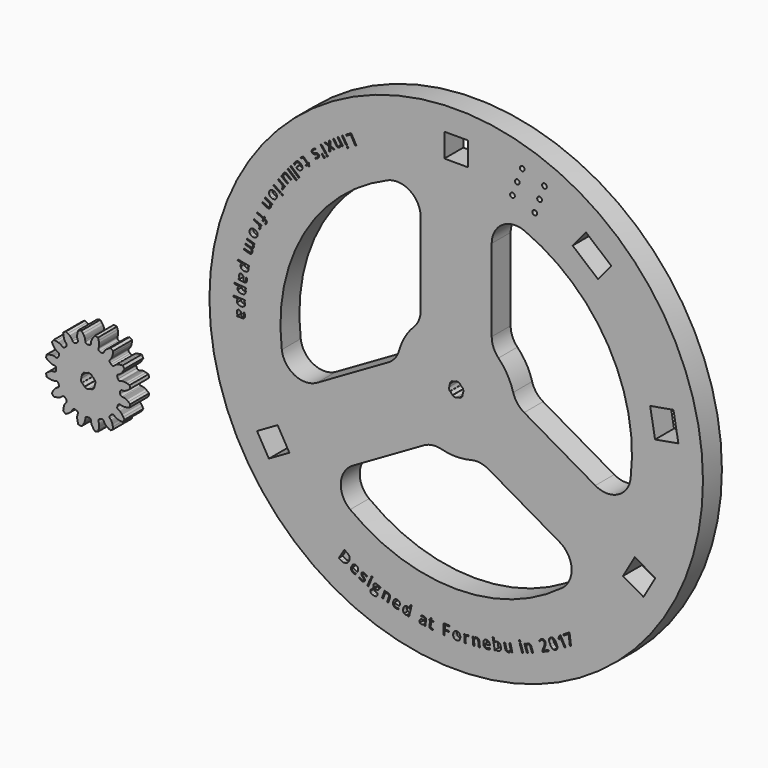
from build123d import *

# Parameters (mm, degrees)
F0_R     = 104.25
F0_R_2   = 1
F0_W     = 10
F0_H     = 10
F1_DEPTH = 10
F3_DEPTH = 2


# Not quite as in the source:
# - ends of sketch curves that miss each other by under 0.0002 mm in the source are joined


with BuildPart() as f1:
    # F0 (on Front) → F1 (new body)
    with BuildSketch(Plane.XZ):
        Circle(F0_R)
        Polygon((-75.46264, -37.794873), (-70.46264, -46.455127), (-79.122894, -51.455127), (-84.122894, -42.794873), align=None, mode=Mode.SUBTRACT)
        with BuildLine():
            ThreePointArc((-44.7894080773, -59.2196881022), (-48.7379690609, -50.6246747393), (-43.7571640164, -42.5837189716))
            Line((-43.7571640164, -42.5837189716), (-13.713203, -25.23783))
            ThreePointArc((-13.713203, -25.23783), (-10.0690355129, -23.9904244279), (-6.2237170045, -24.2129170175))
            ThreePointArc((-6.2237170045, -24.2129170175), (0, -25), (6.2237169853, -24.212916943))
            ThreePointArc((6.2237169853, -24.212916943), (10.0690355129, -23.9904244279), (13.7132030164, -25.2378299716))
            Line((13.7132030164, -25.2378299716), (43.757164, -42.583719))
            ThreePointArc((43.757164, -42.583719), (48.7379690609, -50.6246747393), (44.7894080773, -59.2196881022))
            ThreePointArc((44.7894080773, -59.2196881022), (0, -74.25), (-44.7894080773, -59.2196881022))
        make_face(mode=Mode.SUBTRACT)
        with BuildLine():
            ThreePointArc((-2.6846788138, -1.5499998925), (-2.9943700776, -0.8023389799), (-3.1, 0))
            Line((-3.1, 0), (-2.9, 0))
            ThreePointArc((-2.9, 0), (-2.8011849175, 0.7505751513), (-2.5114737532, 1.4499998575))
            Line((-2.5114737532, 1.4499998575), (-2.684679, 1.55))
            ThreePointArc((-2.684679, 1.55), (-2.1920310217, 2.1920310217), (-1.5499998925, 2.6846788138))
            Line((-1.5499998925, 2.6846788138), (-1.45, 2.511474))
            ThreePointArc((-1.45, 2.511474), (-0.7505751513, 2.8011849175), (0, 2.9))
            Line((0, 2.9), (0, 3.1))
            ThreePointArc((0, 3.1), (0.8023389799, 2.9943700776), (1.5499998925, 2.6846788138))
            Line((1.5499998925, 2.6846788138), (1.45, 2.511474))
            ThreePointArc((1.45, 2.511474), (2.0506096654, 2.0506096654), (2.5114737532, 1.4499998575))
            Line((2.5114737532, 1.4499998575), (2.684679, 1.55))
            ThreePointArc((2.684679, 1.55), (2.9943700776, 0.8023389799), (3.1, 0))
            Line((3.1, 0), (2.9, 0))
            ThreePointArc((2.9, 0), (2.8011849175, -0.7505751513), (2.5114737532, -1.4499998575))
            Line((2.5114737532, -1.4499998575), (2.684679, -1.55))
            ThreePointArc((2.684679, -1.55), (2.1920310217, -2.1920310217), (1.5499998925, -2.6846788138))
            Line((1.5499998925, -2.6846788138), (1.45, -2.511474))
            ThreePointArc((1.45, -2.511474), (0.7505751513, -2.8011849175), (0, -2.9))
            Line((0, -2.9), (0, -3.1))
            ThreePointArc((0, -3.1), (-0.8023389799, -2.9943700776), (-1.5499998925, -2.6846788138))
            Line((-1.5499998925, -2.6846788138), (-1.45, -2.511474))
            ThreePointArc((-1.45, -2.511474), (-2.0506096654, -2.0506096654), (-2.5114737532, -1.4499998575))
            Line((-2.5114737532, -1.4499998575), (-2.6846788138, -1.5499998925))
        make_face(mode=Mode.SUBTRACT)
        Polygon((79.122894, -51.455127), (70.46264, -46.455127), (75.46264, -37.794873), (84.122894, -42.794873), align=None, mode=Mode.SUBTRACT)
        with BuildLine():
            ThreePointArc((-28.8910508851, 68.398608728), (-19.4732699022, 67.520656907), (-15, 59.186675))
            Line((-15, 59.186675), (-15, 24.494897))
            ThreePointArc((-15, 24.494897), (-15.7417990047, 20.715252264), (-17.857142866, 17.4963548687))
            ThreePointArc((-17.857142866, 17.4963548687), (-21.6506351291, 12.4999999402), (-24.0808595484, 6.7165618741))
            ThreePointArc((-24.0808595484, 6.7165618741), (-25.8108340101, 3.275171285), (-28.7132029836, 0.7429319716))
            Line((-28.7132029836, 0.7429319716), (-58.757164, -16.602956))
            ThreePointArc((-58.757164, -16.602956), (-68.2112385185, -16.8959818562), (-73.6804579392, -9.1789209924))
            ThreePointArc((-73.6804579392, -9.1789209924), (-64.3023863966, 37.1249997132), (-28.8910508851, 68.398608728))
        make_face(mode=Mode.SUBTRACT)
        with BuildLine():
            ThreePointArc((17.857142866, 17.4963548687), (15.7417990047, 20.715252264), (15, 24.494897))
            Line((15, 24.494897), (15, 59.186675))
            ThreePointArc((15, 59.186675), (19.4732699022, 67.520656907), (28.8910508851, 68.398608728))
            ThreePointArc((28.8910508851, 68.398608728), (64.3023863966, 37.1249997132), (73.6804581215, -9.1789210151))
            ThreePointArc((73.6804581215, -9.1789210151), (68.2112385185, -16.8959818562), (58.7571639836, -16.6029560284))
            Line((58.7571639836, -16.6029560284), (28.713203, 0.742932))
            ThreePointArc((28.713203, 0.742932), (25.8108340101, 3.275171285), (24.0808590458, 6.7165617338))
            ThreePointArc((24.0808590458, 6.7165617338), (21.6506351291, 12.4999999402), (17.857142866, 17.4963548687))
        make_face(mode=Mode.SUBTRACT)
        Polygon((84.011942, 8.721012), (81.928164, 20.538705), (91.776242, 22.275187), (93.86002, 10.457494), align=None, mode=Mode.SUBTRACT)
        with Locations((33.17164, 76.51931)):
            Circle(F0_R_2, mode=Mode.SUBTRACT)
        with Locations((0, 89.25)):
            Rectangle(F0_W, F0_H, mode=Mode.SUBTRACT)
        with Locations((23.774714, 79.939511)):
            Circle(F0_R_2, mode=Mode.SUBTRACT)
        with Locations((25.826835, 85.577667)):
            Circle(F0_R_2, mode=Mode.SUBTRACT)
        with Locations((27.878956, 91.215823)):
            Circle(F0_R_2, mode=Mode.SUBTRACT)
        Polygon((65.559371, 67.240549), (59.90284, 60.499358), (49.178218, 69.498384), (54.834749, 76.239575), align=None, mode=Mode.SUBTRACT)
        with Locations((35.223761, 82.157466)):
            Circle(F0_R_2, mode=Mode.SUBTRACT)
        with Locations((37.275882, 87.795621)):
            Circle(F0_R_2, mode=Mode.SUBTRACT)
    extrude(amount=-F1_DEPTH)

    # F2 (on Front) → F3 (cut)
    with BuildSketch(Plane.XZ):
        Polygon((-46.5270597802, 79.6829258797), (-46.2968177802, 79.2736728797), (-44.5815277802, 80.2386788797), (-42.6247117802, 76.7604518797), (-42.1729157802, 77.0146278797), (-44.3599747802, 80.9021068797), align=None)
        Polygon((48.4953402198, -79.5741021203), (47.9167592198, -75.1663181203), (47.7033802198, -74.8207741203), (45.1782492198, -76.3800871203), (45.4234312198, -76.7771311203), (47.4917122198, -75.4999301203), (48.0177252198, -79.8690381203), align=None)
        Polygon((-67.2906587802, 56.0793108797), (-70.9337917802, 59.1233418797), (-71.2586637802, 58.7345318797), (-67.6155297802, 55.6904998797), align=None)
        Polygon((30.8113362198, -84.4546881203), (30.2314092198, -84.5637631203), (29.9661432198, -84.6859961203), (29.6878092198, -84.9014401203), (29.5250872198, -85.1092081203), (29.4044442198, -85.4087701203), (29.3814462198, -85.4169411203), (29.1508792198, -85.0129631203), (28.7626802198, -85.1508971203), (29.8821642198, -88.3015591203), (30.3595932198, -88.1319211203), (29.7722322198, -86.4788581203), (29.6482792198, -85.9888821203), (29.6885882198, -85.5144981203), (29.8769042198, -85.2410011203), (30.3175992198, -84.9900311203), (30.6215812198, -84.9234401203), (30.9347362198, -84.9846941203), (31.1278012198, -85.1467861203), (31.3140992198, -85.4969061203), (32.0384132198, -87.5354081203), (32.5158422198, -87.3657691203), (31.7856442198, -85.3107091203), (31.5637012198, -84.8624801203), (31.1858642198, -84.5338861203), align=None)
        Polygon((-53.6710707802, 75.0725808797), (-53.6370527802, 73.4203638797), (-55.1926687802, 73.9630348797), (-55.6556957802, 73.6253978797), (-53.6590157802, 72.9633448797), (-53.6367567802, 70.9594148797), (-53.1753077802, 71.2959018797), (-53.2200387802, 72.8484828797), (-51.7530987802, 72.3329738797), (-51.2869167802, 72.6729128797), (-53.1881007802, 73.3067338797), (-53.2080447802, 75.4102188797), align=None)
        Polygon((-4.8564847802, -91.1642601203), (-3.0096037802, -91.2529211203), (-2.9875087802, -90.7926641203), (-4.8343897802, -90.7040021203), (-4.7561197802, -89.0735991203), (-2.7902747802, -89.1679721203), (-2.7681787802, -88.7077141203), (-5.2518137802, -88.5884841203), (-5.4656977802, -93.0438151203), (-4.9479087802, -93.0686721203), align=None)
        Polygon((-66.1750817802, 57.3825718797), (-69.7583817802, 60.4968138797), (-70.0907477802, 60.1143888797), (-66.5074467802, 57.0001468797), align=None)
        Polygon((39.0197222198, -84.1350671203), (36.9252062198, -85.0711461203), (36.9152482198, -85.0488631203), (37.4169632198, -83.7788571203), (37.6572392198, -83.1064101203), (37.8016072198, -82.4574491203), (37.8011342198, -82.0556711203), (37.6765162198, -81.5937531203), (37.4360192198, -81.2249351203), (36.9980292198, -80.9501121203), (36.5732112198, -80.8981271203), (35.9670292198, -81.0585491203), (35.4434732198, -81.4012201203), (34.9506382198, -82.0741781203), (35.3363522198, -82.2792601203), (35.4964452198, -82.0069611203), (35.7058792198, -81.7494791203), (35.8851862198, -81.6003501203), (36.1488372198, -81.4509981203), (36.4446872198, -81.3630791203), (36.7831112198, -81.3963601203), (37.0056612198, -81.5297371203), (37.2120082198, -81.8248751203), (37.2850752198, -82.0288971203), (37.3268132198, -82.2911101203), (37.3229192198, -82.5071601203), (37.2770792198, -82.8078911203), (37.1830042198, -83.1395611203), (36.9473732198, -83.8048051203), (36.3567412198, -85.3615591203), (36.5347952198, -85.7599631203), (39.2113192198, -84.5637751203), align=None)
        Polygon((-80.9430207802, 36.7048648797), (-80.6576147802, 36.5455888797), (-80.4433807802, 36.3263818797), (-80.3862717802, 36.1358168797), (-80.4456467802, 35.8612498797), (-80.5447667802, 35.6879948797), (-80.7391257802, 35.4457078797), (-80.4242497802, 35.1573438797), (-80.2347437802, 35.3969928797), (-80.0690927802, 35.6799548797), (-79.9797457802, 36.4515038797), (-80.7444217802, 37.1711638797), (-80.9132017802, 37.2480958797), (-80.8324017802, 37.8678678797), (-81.0402677802, 37.9626158797), (-81.2880707802, 37.4189668797), (-83.9725597802, 38.6425958797), (-84.1827067802, 38.1815608797), (-81.4982177802, 36.9579308797), (-81.8512967802, 36.1833208797), (-81.4933057802, 36.0201428797), (-81.1402267802, 36.7947538797), align=None)
        Polygon((-72.6054287802, 57.0290238797), (-73.0378267802, 56.6216288797), (-73.2000517802, 56.3718708797), (-73.3216317802, 56.0433378797), (-73.3477387802, 55.7852488797), (-73.2882027802, 55.4704668797), (-73.3049947802, 55.4488968797), (-73.7035527802, 55.6663908797), (-73.9602287802, 55.3366918797), (-71.3218677802, 53.2826798797), (-71.0106177802, 53.6824778797), (-72.3972017802, 54.7619588797), (-72.7643267802, 55.1071748797), (-72.9875987802, 55.5284228797), (-72.9782367802, 55.8606038797), (-72.7423157802, 56.3099128797), (-72.5223497802, 56.5290788797), (-72.2259017802, 56.6458708797), (-71.9760737802, 56.6131518797), (-71.6302037802, 56.4177978797), (-69.9185427802, 55.0852388797), (-69.6036937802, 55.4896588797), (-71.3299907802, 56.8336128797), (-71.7556087802, 57.0905918797), (-72.2480097802, 57.1641528797), align=None)
        Polygon((44.0685272198, -77.0183181203), (43.6964632198, -77.2270571203), (43.1137302198, -78.6006171203), (43.5179152198, -78.7723601203), (43.7352192198, -78.2215791203), (43.8597982198, -77.8982851203), (43.8885952198, -77.8128891203), (43.9188502198, -77.7112391203), (44.0605662198, -77.9980771203), (44.2648892198, -78.3779111203), (45.8201632198, -81.1500861203), (46.2509742198, -80.9083881203), align=None)
        Polygon((-49.6840267802, 73.7969818797), (-49.1465797802, 74.0406278797), (-48.9179207802, 74.2223468797), (-48.6986967802, 74.4977148797), (-48.5899577802, 74.7381748797), (-48.5438877802, 75.0578158797), (-48.5234877802, 75.0712138797), (-48.2035987802, 74.7335298797), (-47.8592497802, 74.9596878797), (-49.6947717802, 77.7544638797), (-50.1182727802, 77.4763218797), (-49.1552257802, 76.0099828797), (-48.9184847802, 75.5634468797), (-48.8450097802, 75.0930578797), (-48.9630057802, 74.7826698797), (-49.3315117802, 74.4342428797), (-49.6109917802, 74.2973838797), (-49.9297347802, 74.2825338797), (-50.1557647802, 74.3941518797), (-50.4198627802, 74.6900298797), (-51.6074597802, 76.4982698797), (-52.0309597802, 76.2201278797), (-50.8337167802, 74.3971998797), (-50.5116987802, 74.0144828797), (-50.0666487802, 73.7849928797), align=None)
        Polygon((-46.1297967802, 76.0205628797), (-47.8661107802, 78.8780318797), (-48.2991117802, 78.6149228797), (-46.5627977802, 75.7574538797), align=None)
        Polygon((4.1304882198, -90.0705931203), (3.9137742198, -90.3996411203), (3.8893952198, -90.4007881203), (3.8018122198, -89.7852831203), (3.3844412198, -89.8049091203), (3.5414962198, -93.1448571203), (4.0476082198, -93.1210581203), (3.9633252198, -91.3287011203), (4.0001912198, -90.9256791203), (4.2124582198, -90.4955451203), (4.4778322198, -90.2566601203), (4.8903252198, -90.1338231203), (5.0398712198, -90.1356841203), (5.2581682198, -90.1624601203), (5.3063242198, -89.6901031203), (5.1409302198, -89.6723881203), (4.9057382198, -89.6718011203), (4.6410322198, -89.7185901203), (4.3377372198, -89.8758951203), align=None)
        Polygon((27.3079482198, -85.6194751203), (26.8247982198, -85.7720591203), (27.8317362198, -88.9604741203), (28.3148862198, -88.8078901203), align=None)
        Polygon((-46.0898887802, -75.6938961203), (-47.2571907802, -74.9829861203), (-49.5772957802, -78.7925571203), (-48.5217217802, -79.4354231203), (-47.7038967802, -79.8010511203), (-46.7445067802, -79.8336711203), (-46.0733137802, -79.5225851203), (-45.3543337802, -78.7034221203), (-45.0221397802, -77.9434021203), (-45.0085727802, -77.0274051203), (-45.3127797802, -76.3788401203), align=None)
        Polygon((-48.3620177802, -79.0080291203), (-48.9014777802, -78.6794871203), (-47.0480347802, -75.6361661203), (-46.4043507802, -76.0281821203), (-46.2006767802, -76.1633621203), (-46.0225577802, -76.3052551203), (-45.8699917802, -76.4538631203), (-45.7481997802, -76.6019781203), (-45.6496917802, -76.7562111203), (-45.5744667802, -76.9165611203), (-45.5225267802, -77.0830291203), (-45.4931707802, -77.2636381203), (-45.4895367802, -77.4502691203), (-45.5116257802, -77.6429201203), (-45.5567057802, -77.8324321203), (-45.6252237802, -78.0274301203), (-45.7171777802, -78.2279141203), (-45.8325697802, -78.4338841203), (-45.9725557802, -78.6444201203), (-46.1199297802, -78.8284491203), (-46.2746917802, -78.9859731203), (-46.4293107802, -79.1116101203), (-46.5906627802, -79.2130961203), (-46.7587457802, -79.2904321203), (-46.9335607802, -79.3436161203), (-47.1235767802, -79.3731471203), (-47.3202917802, -79.3756071203), (-47.5237077802, -79.3509971203), (-47.7241287802, -79.3022531203), (-47.9306537802, -79.2288441203), (-48.1432827802, -79.1307691203), align=None, mode=Mode.SUBTRACT)
        Polygon((-73.0669027802, 51.9333988797), (-73.0527737802, 51.9532988797), (-72.5141907802, 51.6427438797), (-72.2722987802, 51.9834378797), (-74.9986497802, 53.9191368797), (-75.2919717802, 53.5060048797), (-73.8288957802, 52.4672268797), (-73.5343307802, 52.1897078797), (-73.3265697802, 51.7573798797), (-73.3021217802, 51.4011598797), (-73.4597487802, 51.0006688797), (-73.5534217802, 50.8840798797), (-73.7090997802, 50.7287258797), (-73.3669087802, 50.3995678797), (-73.2509837802, 50.5188588797), (-73.1055067802, 50.7036618797), (-72.9791307802, 50.9409118797), (-72.9159697802, 51.2766838797), (-72.9414677802, 51.5598968797), align=None)
        Polygon((21.6026092198, -90.6491161203), (22.1943972198, -90.5969001203), (22.4764222198, -90.5012051203), (22.7753012198, -90.3184841203), (22.9555932198, -90.1319731203), (23.1037302198, -89.8479171203), (23.1302712198, -89.8413751203), (23.3085992198, -90.2589281203), (23.7142902198, -90.1589331203), (22.9140992198, -86.9124561203), (22.4221512198, -87.0337121203), (22.8426892198, -88.7398891203), (22.9172582198, -89.2382811203), (22.8317862198, -89.7073171203), (22.6187712198, -89.9623801203), (22.1553272198, -90.1691541203), (21.8468982198, -90.2050761203), (21.5417902198, -90.1132531203), (21.3658592198, -89.9328851203), (21.2151992198, -89.5653381203), (20.6960682198, -87.4591561203), (20.1984332198, -87.5818131203), (20.7220032198, -89.7060041203), (20.8971352198, -90.1713191203), (21.2382702198, -90.5339441203), align=None)
        Polygon((-78.3656857802, 42.1996808797), (-78.2491517802, 42.4674988797), (-78.1849267802, 42.8135648797), (-78.2018527802, 43.0769258797), (-78.3112907802, 43.3807608797), (-78.2995727802, 43.4021698797), (-77.8585687802, 43.2542698797), (-77.6607647802, 43.6156528797), (-80.5937887802, 45.2210468797), (-80.8370587802, 44.7765968797), (-79.2981847802, 43.9342928797), (-78.8794677802, 43.6512428797), (-78.5936917802, 43.2704588797), (-78.5520987802, 42.9410138797), (-78.7138087802, 42.4603398797), (-78.8962777802, 42.2082598797), (-79.1707117802, 42.0454588797), (-79.4226847802, 42.0378528797), (-79.7947997802, 42.1750438797), (-81.6924877802, 43.2137458797), (-81.9357567802, 42.7692958797), (-80.0226557802, 41.7221568797), (-79.5586217802, 41.5354988797), (-79.0579287802, 41.5418988797), (-78.7257547802, 41.7321738797), align=None)
        Polygon((-64.3416257802, 64.8230158797), (-62.9564677802, 63.4248768797), (-63.6458287802, 62.7419178797), (-63.3689347802, 62.4624278797), (-62.6795737802, 63.1453878797), (-62.1340307802, 62.5947318797), (-61.9259747802, 62.8008568797), (-62.2770437802, 63.4576048797), (-62.0849347802, 63.9447628797), (-62.2567047802, 64.1181428797), (-62.5972237802, 63.7807858797), (-63.9974977802, 65.1941818797), (-64.6246027802, 65.5605008797), (-65.4055387802, 65.2380268797), (-65.4868037802, 65.1503328797), (-65.5922697802, 65.0159248797), (-65.6635637802, 64.9091838797), (-65.7182287802, 64.7990628797), (-65.4454577802, 64.5237348797), (-65.4056047802, 64.5892898797), (-65.3335297802, 64.6923408797), (-65.2635017802, 64.7805838797), (-65.1627947802, 64.8889748797), (-64.9991787802, 65.0070408797), (-64.7695937802, 65.0510908797), (-64.5804617802, 65.0001468797), align=None)
        Polygon((27.1046632198, -84.9057001203), (27.0816652198, -84.7408771203), (27.0252302198, -84.6189771203), (26.9211242198, -84.5259091203), (26.8237162198, -84.4972931203), (26.6956682198, -84.5106031203), (26.6002762198, -84.5571791203), (26.5157312198, -84.6524011203), (26.4867012198, -84.7551751203), (26.5110092198, -84.9210971203), (26.5669882198, -85.0434391203), (26.6691982198, -85.1383441203), (26.7662542198, -85.1681261203), (26.8988192198, -85.1538711203), (26.9901082198, -85.1079961203), (27.0741502198, -85.0104551203), align=None)
        Polygon((-82.9995267802, 34.0885308797), (-82.9902547802, 34.1111068797), (-82.3954677802, 33.9301498797), (-82.2367297802, 34.3166558797), (-85.3296767802, 35.5869288797), (-85.5221657802, 35.1182458797), (-83.8623587802, 34.4365638797), (-83.5127487802, 34.2327048797), (-83.2127557802, 33.8584368797), (-83.1085247802, 33.5169318797), (-83.1716737802, 33.0911948797), (-83.2366087802, 32.9564698797), (-83.3531987802, 32.7699828797), (-82.9455347802, 32.5265688797), (-82.8595317802, 32.6689498797), (-82.7595277802, 32.8818228797), (-82.6899717802, 33.1414768797), (-82.7042397802, 33.4828408797), (-82.7930137802, 33.7529858797), align=None)
        Polygon((9.0766592198, -89.4424411203), (8.4877732198, -89.4046841203), (8.2005162198, -89.4575081203), (7.8775412198, -89.5974131203), (7.6684862198, -89.7584761203), (7.4774962198, -90.0188901203), (7.4531922198, -90.0211191203), (7.3297112198, -89.5726641203), (6.9194572198, -89.6102931203), (7.2248572198, -92.9399551203), (7.7294102198, -92.8936771203), (7.5691762198, -91.1466981203), (7.5702672198, -90.6412881203), (7.7266602198, -90.1916151203), (7.9767732198, -89.9731951203), (8.4658502198, -89.8390261203), (8.7768572198, -89.8496931203), (9.0651312198, -89.9865001203), (9.2121052198, -90.1913091203), (9.3060142198, -90.5766301203), (9.5036092198, -92.7309461203), (10.0081622198, -92.6846681203), (9.8089622198, -90.5128531203), (9.7047812198, -90.0236551203), (9.4199612198, -89.6118151203), align=None)
        Polygon((-54.8354537802, 70.0295188797), (-56.8961647802, 72.6626508797), (-57.2951707802, 72.3503848797), (-55.2344597802, 69.7172528797), align=None)
        Polygon((-10.7706187802, -91.8718711203), (-10.7809197802, -91.5746981203), (-10.5506257802, -89.6201091203), (-9.5869047802, -89.7336561203), (-9.5408687802, -89.3429331203), (-10.5045897802, -89.2293851203), (-10.4138887802, -88.4595711203), (-10.7047497802, -88.4253011203), (-10.9996137802, -89.1091311203), (-11.5003317802, -89.2624631203), (-11.5288897802, -89.5048471203), (-11.0528467802, -89.5609361203), (-11.2856537802, -91.5368551203), (-11.1813607802, -92.2555851203), (-10.4425047802, -92.6653951203), (-10.3232797802, -92.6743041203), (-10.1524367802, -92.6730311203), (-10.0245277802, -92.6622711203), (-9.9043377802, -92.6364011203), (-9.8589877802, -92.2514951203), (-9.9350927802, -92.2611781203), (-10.0606017802, -92.2690261203), (-10.1732557802, -92.2692471203), (-10.3207837802, -92.2580311203), (-10.5150807802, -92.2036421203), (-10.6926017802, -92.0515361203), align=None)
        Polygon((-47.0480347802, -75.6361661203), (-48.9014777802, -78.6794871203), (-48.3620177802, -79.0080291203), (-48.1432827802, -79.1307691203), (-47.9306537802, -79.2288441203), (-47.7241287802, -79.3022531203), (-47.5237077802, -79.3509971203), (-47.3202917802, -79.3756071203), (-47.1235767802, -79.3731471203), (-46.9335607802, -79.3436161203), (-46.7587457802, -79.2904321203), (-46.5906627802, -79.2130961203), (-46.4293107802, -79.1116101203), (-46.2746917802, -78.9859731203), (-46.1199297802, -78.8284491203), (-45.9725557802, -78.6444201203), (-45.8325697802, -78.4338841203), (-45.7171777802, -78.2279141203), (-45.6252237802, -78.0274301203), (-45.5567057802, -77.8324321203), (-45.5116257802, -77.6429201203), (-45.4895367802, -77.4502691203), (-45.4931707802, -77.2636381203), (-45.5225267802, -77.0830291203), (-45.5744667802, -76.9165611203), (-45.6496917802, -76.7562111203), (-45.7481997802, -76.6019781203), (-45.8699917802, -76.4538631203), (-46.0225577802, -76.3052551203), (-46.2006767802, -76.1633621203), (-46.4043507802, -76.0281821203), align=None)
        Polygon((-86.0940327802, 22.9863558797), (-86.0381677802, 23.2868208797), (-86.0616197802, 23.6501278797), (-86.1492817802, 23.9080988797), (-86.3407747802, 24.1812408797), (-86.3340127802, 24.2046918797), (-85.8713717802, 24.4014838797), (-85.5040497802, 25.0321738797), (-85.4541867802, 25.3012518797), (-85.4744097802, 25.6317188797), (-85.5532267802, 25.8699188797), (-85.7290487802, 26.1262968797), (-85.7222857802, 26.1497478797), (-85.2596327802, 26.1016718797), (-85.1454767802, 26.4975158797), (-88.3581887802, 27.4240128797), (-88.4985837802, 26.9371818797), (-86.8129657802, 26.4510748797), (-86.3429927802, 26.2709888797), (-85.9756147802, 25.9794648797), (-85.8551697802, 25.6909738797), (-85.8947227802, 25.2311998797), (-86.0100967802, 24.9706158797), (-86.2345167802, 24.7734238797), (-86.4731347802, 24.7201918797), (-86.8582677802, 24.7754988797), (-88.9481717802, 25.3781958797), (-89.0885667802, 24.8913648797), (-87.2941387802, 24.3738778797), (-86.8836287802, 24.2099568797), (-86.5538177802, 23.9251698797), (-86.4431577802, 23.6366048797), (-86.4865987802, 23.1788168797), (-86.6014167802, 22.9201638797), (-86.8255817802, 22.7238538797), (-87.0641997802, 22.6706228797), (-87.4493327802, 22.7259298797), (-89.5392367802, 23.3286258797), (-89.6793617802, 22.8427328797), (-87.5838287802, 22.2384128797), (-87.0914727802, 22.1532718797), (-86.6093757802, 22.2510278797), (-86.3330957802, 22.4871868797), align=None)
        Polygon((-58.6446007802, 67.3696408797), (-58.9566477802, 67.1523948797), (-59.4693467802, 66.9291508797), (-59.3361597802, 66.4994958797), (-58.8904917802, 66.6860178797), (-58.3938887802, 67.0249828797), (-58.0748017802, 67.3619648797), (-57.8596237802, 67.8008738797), (-57.8451217802, 68.1331638797), (-58.0307567802, 68.5069718797), (-58.1683327802, 68.6373868797), (-58.3606907802, 68.7410468797), (-58.5297487802, 68.7772558797), (-58.7747727802, 68.7718048797), (-59.0255007802, 68.7170638797), (-59.4749807802, 68.5670288797), (-59.8576657802, 68.4430768797), (-60.1893217802, 68.3822988797), (-60.3639927802, 68.4069068797), (-60.5355667802, 68.5241118797), (-60.6370657802, 68.7043878797), (-60.6270947802, 68.9556218797), (-60.5152227802, 69.1673078797), (-60.2490067802, 69.4503168797), (-60.0665807802, 69.5904328797), (-59.8007537802, 69.7461928797), (-59.5755367802, 69.8466088797), (-59.2844187802, 69.9395978797), (-59.5918347802, 70.2945548797), (-59.9768747802, 70.1525618797), (-60.5135947802, 69.7752088797), (-60.8585547802, 69.4115688797), (-61.0857007802, 68.9445908797), (-61.0930417802, 68.5886798797), (-60.8770627802, 68.1728208797), (-60.6690557802, 67.9944258797), (-60.3573987802, 67.8919088797), (-60.0358197802, 67.9154548797), (-59.4643737802, 68.0880368797), (-59.1335367802, 68.2055318797), (-58.8595837802, 68.2844358797), (-58.7201657802, 68.3034858797), (-58.5748377802, 68.2934118797), (-58.4797187802, 68.2557438797), (-58.3729387802, 68.1654188797), (-58.2963807802, 68.0228918797), (-58.3077467802, 67.8105448797), (-58.4047707802, 67.6241278797), align=None)
        Polygon((-56.5445617802, 69.3012308797), (-56.7928507802, 69.0990288797), (-55.8702957802, 67.7729548797), (-55.4304907802, 68.1311238797), align=None)
        Polygon((-74.1624497802, 49.2643978797), (-76.9444607802, 51.1192098797), (-77.2255257802, 50.6976438797), (-74.4435147802, 48.8428318797), align=None)
        Polygon((-28.2185557802, -85.2915671203), (-28.7400187802, -85.0153631203), (-29.0236357802, -84.9455911203), (-29.3755747802, -84.9405591203), (-29.6323247802, -85.0015901203), (-29.9133927802, -85.1606291203), (-29.9364687802, -85.1526831203), (-29.8649427802, -84.6930711203), (-30.2544737802, -84.5589461203), (-31.3430467802, -87.7204211203), (-30.8639797802, -87.8853761203), (-30.2928357802, -86.2266401203), (-30.0843367802, -85.7662401203), (-29.7571117802, -85.4204231203), (-29.4393757802, -85.3239491203), (-28.9383347802, -85.4024081203), (-28.6591287802, -85.5398241203), (-28.4524397802, -85.7829241203), (-28.4025117802, -86.0300181203), (-28.4750827802, -86.4199211203), (-29.1793977802, -88.4654191203), (-28.7003307802, -88.6303731203), (-27.9902947802, -86.5682611203), (-27.8844417802, -86.0794221203), (-27.9750627802, -85.5869561203), align=None)
        Polygon((-46.1955957802, 75.1125028797), (-46.1340597802, 74.9578778797), (-46.0502537802, 74.8528958797), (-45.9270017802, 74.7872568797), (-45.8255827802, 74.7826268797), (-45.7043737802, 74.8260078797), (-45.6227947802, 74.8939338797), (-45.5633217802, 75.0065308797), (-45.5595657802, 75.1132598797), (-45.6226357802, 75.2686408797), (-45.7061047802, 75.3741588797), (-45.8279517802, 75.4420338797), (-45.9293057802, 75.4478798797), (-46.0546777802, 75.4025068797), (-46.1324377802, 75.3362378797), (-46.1908707802, 75.2215088797), align=None)
        Polygon((14.0240572198, -92.1107661203), (14.2974302198, -91.9621741203), (14.2340842198, -91.5146331203), (13.7940112198, -91.7332561203), (13.2091832198, -91.8874591203), (12.7984962198, -91.8859361203), (12.3796082198, -91.6967601203), (12.1395492198, -91.4041431203), (11.9595382198, -90.8535571203), (14.2397712198, -90.5308111203), (14.1948962198, -90.2137631203), (14.0483292198, -89.6839871203), (13.6795262198, -89.1848811203), (13.2706222198, -88.9561441203), (12.6375762198, -88.9147991203), (12.1176622198, -89.0814451203), (11.6448692198, -89.5359711203), (11.4419072198, -90.0528691203), (11.4306082198, -90.8643341203), (11.6022182198, -91.4840551203), (12.0311042198, -92.0453311203), (12.5082202198, -92.2911461203), (13.2529322198, -92.3288991203), (13.5276312198, -92.2800921203), (13.8180512198, -92.1976411203), align=None)
        Polygon((13.6223042198, -90.0712761203), (13.6446002198, -90.1989701203), (11.9134012198, -90.4440061203), (11.9116112198, -90.3112601203), (11.9194172198, -90.1859151203), (11.9368172198, -90.0679721203), (11.9623772198, -89.9622941203), (11.9966802198, -89.8633601203), (12.0397252198, -89.7711701203), (12.0915132198, -89.6857231203), (12.1545982198, -89.6048331203), (12.2261882198, -89.5341291203), (12.3062832198, -89.4736111203), (12.3906702198, -89.4253451203), (12.4828062198, -89.3863601203), (12.5826912198, -89.3566561203), (12.6903242198, -89.3362331203), (12.8025732198, -89.3258801203), (12.9085202198, -89.3274921203), (13.0081642198, -89.3410661203), (13.0973992198, -89.3651841203), (13.1808912198, -89.4002021203), (13.2586412198, -89.4461211203), (13.3306482198, -89.5029401203), (13.3992062198, -89.5735791203), (13.4600262198, -89.6550281203), (13.5131082198, -89.7472861203), (13.5565572198, -89.8454341203), (13.5929562198, -89.9534301203), align=None, mode=Mode.SUBTRACT)
        Polygon((16.1901542198, -88.5667161203), (16.1201502198, -88.1637061203), (15.9014312198, -87.0307031203), (15.4039452198, -87.1267391203), (16.3038022198, -91.7881561203), (16.6603822198, -91.7193201203), (16.6832602198, -91.2764311203), (16.7196852198, -91.2694001203), (16.9310992198, -91.4277541203), (17.2343802198, -91.5483601203), (17.4941562198, -91.5824971203), (17.8433852198, -91.5535881203), (18.3366722198, -91.3683731203), (18.7590392198, -90.9120061203), (18.9171422198, -90.3999701203), (18.8772502198, -89.5852031203), (18.6843512198, -88.9583841203), (18.2779382198, -88.4043701203), (17.8483792198, -88.1726771203), (17.1875972198, -88.1564961203), (16.6696452198, -88.3550381203), (16.2519002198, -88.8461921203), (16.2279362198, -88.8508181203), align=None)
        Polygon((17.8249562198, -91.1178471203), (17.7025032198, -91.1482771203), (17.5579522198, -91.1695311203), (17.4229042198, -91.1756461203), (17.2973612198, -91.1666231203), (17.1863902198, -91.1438891203), (17.0840792198, -91.1073621203), (16.9904282198, -91.0570421203), (16.9054362198, -90.9929291203), (16.8242562198, -90.9091061203), (16.7497222198, -90.8064191203), (16.6818342198, -90.6848691203), (16.6232312198, -90.5512461203), (16.5706842198, -90.4004361203), (16.5241932198, -90.2324381203), (16.4837572198, -90.0472521203), (16.4510652198, -89.8519191203), (16.4313672198, -89.6719371203), (16.4246632198, -89.5073061203), (16.4303852198, -89.3644771203), (16.4479472198, -89.2356351203), (16.4773492198, -89.1207791203), (16.5185912198, -89.0199111203), (16.5753242198, -88.9266631203), (16.6467092198, -88.8436121203), (16.7327452198, -88.7707591203), (16.8285372198, -88.7107281203), (16.9376802198, -88.6599891203), (17.0601722198, -88.6185411203), (17.1960142198, -88.5863831203), (17.3298272198, -88.5675671203), (17.4557142198, -88.5643111203), (17.5736762198, -88.5766151203), (17.6788822198, -88.6028751203), (17.7768682198, -88.6433141203), (17.8676322198, -88.6979301203), (17.9511752198, -88.7667241203), (18.0314362198, -88.8541861203), (18.1047412198, -88.9575761203), (18.1710902198, -89.0768961203), (18.2279352198, -89.2056521203), (18.2784422198, -89.3489221203), (18.3226102198, -89.5067061203), (18.3604412198, -89.6790041203), (18.3898382198, -89.8572651203), (18.4071402198, -90.0248361203), (18.4123482198, -90.1817171203), (18.4014842198, -90.3659221203), (18.3710282198, -90.5328101203), (18.3209812198, -90.6823821203), (18.2675542198, -90.7868821203), (18.2013112198, -90.8789501203), (18.1222522198, -90.9585841203), (18.0348312198, -91.0230011203), (17.9357322198, -91.0760881203), align=None, mode=Mode.SUBTRACT)
        Polygon((-85.0649567802, 31.7644948797), (-85.4902187802, 31.8782678797), (-85.9963057802, 31.8977538797), (-86.3555647802, 31.8171608797), (-86.7465237802, 31.5966808797), (-86.9927657802, 31.3392688797), (-87.2142467802, 30.9182288797), (-87.3259987802, 30.3439888797), (-87.1665527802, 29.6921278797), (-86.8162397802, 29.2662038797), (-86.1034107802, 28.8730788797), (-85.4772587802, 28.7332438797), (-84.7752147802, 28.8353518797), (-84.3316557802, 29.1217698797), (-83.9589017802, 29.7262488797), (-83.8467757802, 30.2998518797), (-84.0046647802, 30.9490618797), (-84.3534747802, 31.3726658797), align=None)
        Polygon((-86.8589327802, 30.1579138797), (-86.8830237802, 30.2743398797), (-86.8901517802, 30.3900158797), (-86.8817787802, 30.5101278797), (-86.8579067802, 30.6346768797), (-86.8185357802, 30.7636608797), (-86.7642277802, 30.8935318797), (-86.6998417802, 31.0087818797), (-86.6253767802, 31.1094118797), (-86.5448947802, 31.1918298797), (-86.4552307802, 31.2609258797), (-86.3563827802, 31.3167008797), (-86.2483517802, 31.3591548797), (-86.1260337802, 31.3892388797), (-85.9950497802, 31.4044958797), (-85.8554007802, 31.4049258797), (-85.7140157802, 31.3915058797), (-85.5647357802, 31.3645768797), (-85.4075587802, 31.3241368797), (-85.2424867802, 31.2701888797), (-85.0723857802, 31.2033058797), (-84.9189147802, 31.1308158797), (-84.7820727802, 31.0527168797), (-84.6669637802, 30.9729368797), (-84.5670067802, 30.8880468797), (-84.4822017802, 30.7980468797), (-84.4125487802, 30.7029368797), (-84.3558977802, 30.5980638797), (-84.3160107802, 30.4880778797), (-84.2928887802, 30.3729788797), (-84.2864557802, 30.2583408797), (-84.2952977802, 30.1390438797), (-84.3194147802, 30.0150868797), (-84.3588057802, 29.8864718797), (-84.4136637802, 29.7547908797), (-84.4783437802, 29.6378838797), (-84.5528457802, 29.5357518797), (-84.6331247802, 29.4520428797), (-84.7223537802, 29.3817948797), (-84.8205317802, 29.3250088797), (-84.9276607802, 29.2816828797), (-85.0489097802, 29.2507928797), (-85.1788237802, 29.2347948797), (-85.3174017802, 29.2336908797), (-85.4577627802, 29.2465298797), (-85.6060177802, 29.2729388797), (-85.7621667802, 29.3129168797), (-85.9262097802, 29.3664658797), (-86.0959277802, 29.4333108797), (-86.2493277802, 29.5060768797), (-86.3864097802, 29.5847638797), (-86.5020387802, 29.6653978797), (-86.6027997802, 29.7514258797), (-86.6886927802, 29.8428488797), (-86.7597167802, 29.9396678797), (-86.8178307802, 30.0463568797), align=None, mode=Mode.SUBTRACT)
        Polygon((-76.6104697802, 48.5946138797), (-77.0032127802, 48.7934738797), (-77.4944557802, 48.9166978797), (-77.8626107802, 48.9117678797), (-78.2905767802, 48.7764698797), (-78.5845237802, 48.5752458797), (-78.8879167802, 48.2088018797), (-79.1154587802, 47.6698548797), (-79.0935827802, 46.9991328797), (-78.8384257802, 46.5102298797), (-78.2217647802, 45.9788158797), (-77.6377957802, 45.7131078797), (-76.9297667802, 45.6685458797), (-76.4367557802, 45.8575438797), (-75.9475767802, 46.3723678797), (-75.7197997802, 46.9106158797), (-75.7406967802, 47.5784228797), (-75.9948587802, 48.0647458797), align=None)
        Polygon((-77.9468157802, 46.4251718797), (-78.0991427802, 46.5255148797), (-78.2342837802, 46.6282938797), (-78.3522367802, 46.7335088797), (-78.4487957802, 46.8362138797), (-78.5296937802, 46.9411378797), (-78.5949327802, 47.0482808797), (-78.6445107802, 47.1576438797), (-78.6794227802, 47.2740088797), (-78.6966857802, 47.3916378797), (-78.6962997802, 47.5105298797), (-78.6794677802, 47.6251958797), (-78.6465557802, 47.7410138797), (-78.5975617802, 47.8579828797), (-78.5324867802, 47.9761028797), (-78.4526137802, 48.0920168797), (-78.3658867802, 48.1915488797), (-78.2723057802, 48.2746988797), (-78.1765847802, 48.3387888797), (-78.0746187802, 48.3879518797), (-77.9664087802, 48.4221898797), (-77.8519527802, 48.4415008797), (-77.7260617802, 48.4457678797), (-77.5947417802, 48.4337408797), (-77.4579937802, 48.4054218797), (-77.2760997802, 48.3458148797), (-77.0854117802, 48.2598158797), (-76.8859307802, 48.1474258797), (-76.7332357802, 48.0469678797), (-76.5979687802, 47.9444438797), (-76.4801297802, 47.8398538797), (-76.3839037802, 47.7380918797), (-76.3035577802, 47.6344468797), (-76.2390907802, 47.5289198797), (-76.1905027802, 47.4215108797), (-76.1566487802, 47.3072248797), (-76.1402517802, 47.1913838797), (-76.1413127802, 47.0739898797), (-76.1586107802, 46.9604818797), (-76.1918147802, 46.8455578797), (-76.2409267802, 46.7292188797), (-76.3059447802, 46.6114638797), (-76.3867287802, 46.4938918797), (-76.4740837802, 46.3927998797), (-76.5680107802, 46.3081858797), (-76.6637997802, 46.2427908797), (-76.7655757802, 46.1924108797), (-76.8733387802, 46.1570458797), (-76.9870907802, 46.1366958797), (-77.1121027802, 46.1314208797), (-77.2425277802, 46.1425028797), (-77.3783657802, 46.1699418797), (-77.5590807802, 46.2285228797), (-77.7485637802, 46.3135988797), align=None, mode=Mode.SUBTRACT)
        Polygon((-54.7938667802, 69.1200278797), (-54.7145517802, 68.9737248797), (-54.6189667802, 68.8793418797), (-54.4888427802, 68.8286728797), (-54.3875837802, 68.8360178797), (-54.2723257802, 68.8933688797), (-54.1993137802, 68.9704288797), (-54.1535137802, 69.0892448797), (-54.1623507802, 69.1956738797), (-54.2432787802, 69.3425478797), (-54.3385917802, 69.4375038797), (-54.4675837802, 69.4905578797), (-54.5689217802, 69.4844278797), (-54.6880787802, 69.4246078797), (-54.7574937802, 69.3496438797), (-54.8020107802, 69.2288328797), align=None)
        Polygon((39.2630592198, -80.8263301203), (39.6663842198, -81.8734221203), (40.1330282198, -82.6329011203), (40.7763122198, -83.2321211203), (41.3117292198, -83.4102671203), (42.0170502198, -83.2580181203), (42.4896232198, -82.8944921203), (42.7537112198, -82.2446281203), (42.6984752198, -81.5823621203), (42.2975772198, -80.5390411203), (41.8344962198, -79.7872141203), (41.1903172198, -79.1888401203), (40.6513082198, -79.0087591203), (39.9399712198, -79.1623431203), (39.4713212198, -79.5226081203), (39.2080612198, -80.1667551203), align=None)
        Polygon((41.7133032198, -80.5450471203), (41.8343752198, -80.7739481203), (41.9526242198, -81.0179111203), (42.0522092198, -81.2466621203), (42.1331312198, -81.4602011203), (42.1929642198, -81.6498441203), (42.2357922198, -81.8256271203), (42.2616152198, -81.9875491203), (42.2704322198, -82.1356121203), (42.2610172198, -82.2775521203), (42.2321132198, -82.4076671203), (42.1837202198, -82.5259551203), (42.1193452198, -82.6278351203), (42.0372132198, -82.7189401203), (41.9373222198, -82.7992701203), (41.8196742198, -82.8688241203), (41.6897852198, -82.9239831203), (41.5616482198, -82.9568261203), (41.4352612198, -82.9673531203), (41.3162542198, -82.9565861203), (41.1988422198, -82.9254851203), (41.0830252198, -82.8740521203), (40.9688042198, -82.8022871203), (40.8492242198, -82.7040751203), (40.7281322198, -82.5811051203), (40.6055272198, -82.4333791203), (40.4870852198, -82.2692721203), (40.3672652198, -82.0826081203), (40.2460672198, -81.8733851203), (40.1234912198, -81.6416051203), (40.0039302198, -81.3949621203), (39.9035152198, -81.1642971203), (39.8222482198, -80.9496121203), (39.7625352198, -80.7595901203), (39.7202682198, -80.5841281203), (39.6954472198, -80.4232251203), (39.6880722198, -80.2768821203), (39.6989692198, -80.1370161203), (39.7288382198, -80.0087921203), (39.7776792198, -79.8922081203), (39.8419982198, -79.7917831203), (39.9236022198, -79.7019651203), (40.0224942198, -79.6227541203), (40.1386712198, -79.5541491203), (40.2702082198, -79.4982261203), (40.3997132198, -79.4649011203), (40.5271862198, -79.4541751203), (40.6469712198, -79.4650181203), (40.7649052198, -79.4964511203), (40.8809872198, -79.5484751203), (40.9952192198, -79.6210911203), (41.1145632198, -79.7200091203), (41.2351892198, -79.8430481203), (41.3570992198, -79.9902071203), (41.4746642198, -80.1531761203), (41.5933992198, -80.3381231203), align=None, mode=Mode.SUBTRACT)
        Polygon((-39.6099357802, -81.6901601203), (-39.6132647802, -81.5879071203), (-39.5729377802, -81.4539891203), (-39.4726887802, -81.3270031203), (-39.2733827802, -81.2528611203), (-39.0637467802, -81.2676191203), (-38.7347987802, -81.3862611203), (-38.4112517802, -81.5859751203), (-38.0022927802, -81.9673551203), (-37.6612217802, -81.6740771203), (-38.0098017802, -81.3395581203), (-38.5184977802, -81.0190281203), (-38.9546807802, -80.8605391203), (-39.4429767802, -80.8379571203), (-39.7535537802, -80.9569901203), (-40.0225097802, -81.2761371203), (-40.0873467802, -81.4542691203), (-40.1058247802, -81.6719981203), (-40.0717117802, -81.8414911203), (-39.9691317802, -82.0640751203), (-39.8190657802, -82.2722621203), (-39.5024367802, -82.6248081203), (-39.2363347802, -82.9264731203), (-39.0485027802, -83.2064881203), (-39.0015117802, -83.3765101203), (-39.0406927802, -83.5805681203), (-39.1656327802, -83.7454651203), (-39.4000557802, -83.8363731203), (-39.6387827802, -83.8180591203), (-40.0044017802, -83.6865731203), (-40.2055777802, -83.5750391203), (-40.4543177802, -83.3932341203), (-40.6361207802, -83.2266381203), (-40.8373537802, -82.9966351203), (-41.0405197802, -83.4199821203), (-40.7569317802, -83.7166221203), (-40.1970457802, -84.0586621203), (-39.7261057802, -84.2302671203), (-39.2072967802, -84.2526481203), (-38.8779047802, -84.1176411203), (-38.5824597802, -83.7539131203), (-38.5016617802, -83.4920671203), (-38.5317417802, -83.1653641203), (-38.6814097802, -82.8797641203), (-39.0672927802, -82.4243201203), (-39.3068247802, -82.1676431203), (-39.4883027802, -81.9477751203), (-39.5612997802, -81.8274781203), align=None)
        Polygon((-24.3584547802, -89.2991141203), (-24.8494777802, -89.3180041203), (-25.4460977802, -89.2187701203), (-25.8200267802, -89.0489361203), (-26.1244677802, -88.7045961203), (-26.2233877802, -88.3392641203), (-26.1617357802, -87.7632881203), (-23.9497497802, -88.4041841203), (-23.8606387802, -88.0966261203), (-23.7770197802, -87.5533471203), (-23.9086637802, -86.9468881203), (-24.1877747802, -86.5705631203), (-24.7481647802, -86.2732091203), (-25.2906847802, -86.2119481203), (-25.9083057802, -86.4325651203), (-26.3054177802, -86.8207391203), (-26.6485477802, -87.5561741203), (-26.7462177802, -88.1917561203), (-26.5852767802, -88.8795581203), (-26.2509607802, -89.2994361203), (-25.5872567802, -89.6393141203), (-25.3167087802, -89.7074701203), (-25.0180227802, -89.7513901203), (-24.7945097802, -89.7566531203), (-24.4842437802, -89.7332591203), align=None)
        Polygon((-24.3244107802, -87.7318241203), (-24.3564497802, -87.8574291203), (-26.0358337802, -87.3708471203), (-25.9830197802, -87.2490461203), (-25.9244907802, -87.1379311203), (-25.8602467802, -87.0375021203), (-25.7935907802, -86.9516061203), (-25.7217277802, -86.8754451203), (-25.6446577802, -86.8090221203), (-25.5623807802, -86.7523341203), (-25.4716687802, -86.7044361203), (-25.3773777802, -86.6693161203), (-25.2795087802, -86.6469731203), (-25.1827497802, -86.6375651203), (-25.0827297802, -86.6398001203), (-24.9794497802, -86.6536781203), (-24.8729097802, -86.6791981203), (-24.7662907802, -86.7157961203), (-24.6703267802, -86.7607201203), (-24.5850177802, -86.8139691203), (-24.5135257802, -86.8725651203), (-24.4517427802, -86.9387471203), (-24.3996667802, -87.0125151203), (-24.3572997802, -87.0938691203), (-24.3237467802, -87.1864131203), (-24.3016847802, -87.2856411203), (-24.2911127802, -87.3915531203), (-24.2917417802, -87.4988861203), (-24.3028407802, -87.6123101203), align=None, mode=Mode.SUBTRACT)
        Polygon((-1.1853387802, -90.7292121203), (-1.3122757802, -91.5314741203), (-1.2748767802, -91.9701011203), (-1.1213447802, -92.4527311203), (-0.9235427802, -92.7632731203), (-0.5834017802, -93.0561291203), (-0.2576657802, -93.2003251203), (0.2135652198, -93.2656661203), (0.7916302198, -93.1757761203), (1.3506102198, -92.8044431203), (1.6322632198, -92.3303091203), (1.7599622198, -91.5263411203), (1.6788572198, -90.8899121203), (1.3444132198, -90.2642611203), (0.9243902198, -89.9443221203), (0.2292512198, -89.7989901203), (-0.3483417802, -89.8883141203), (-0.9053577802, -90.2572811203), align=None)
        Polygon((1.2303802198, -91.3547371203), (1.2357192198, -91.5272171203), (1.2304802198, -91.7095491203), (1.2141302198, -91.8785431203), (1.1866702198, -92.0342001203), (1.1500942198, -92.1703401203), (1.1033942198, -92.2943271203), (1.0465712198, -92.4061611203), (0.9796252198, -92.5058431203), (0.8990112198, -92.5967331203), (0.8080402198, -92.6732761203), (0.7067132198, -92.7354721203), (0.6003322198, -92.7814571203), (0.4845142198, -92.8143711203), (0.3592602198, -92.8342121203), (0.2245712198, -92.8409811203), (0.0839762198, -92.8340021203), (-0.0462907802, -92.8125791203), (-0.1662277802, -92.7767121203), (-0.2710777802, -92.7290011203), (-0.3665167802, -92.6681281203), (-0.4525447802, -92.5940941203), (-0.5291607802, -92.5069001203), (-0.5989947802, -92.4020661203), (-0.6578247802, -92.2840471203), (-0.7056527802, -92.1528431203), (-0.7410417802, -92.0153021203), (-0.7664057802, -91.8657481203), (-0.7817437802, -91.7041791203), (-0.7870567802, -91.5305961203), (-0.7819127802, -91.3478911203), (-0.7658457802, -91.1789231203), (-0.7388577802, -91.0236921203), (-0.7029077802, -90.8883311203), (-0.6570057802, -90.7654861203), (-0.6011517802, -90.6551581203), (-0.5353467802, -90.5573471203), (-0.4559437802, -90.4684491203), (-0.3660387802, -90.3935831203), (-0.2656307802, -90.3327491203), (-0.1599897802, -90.2877691203), (-0.0447787802, -90.2555751203), (0.0800012198, -90.2361651203), (0.2143502198, -90.2295401203), (0.3568342198, -90.2364211203), (0.4887582198, -90.2575581203), (0.6101222198, -90.2929501203), (0.7161182198, -90.3400321203), (0.8124912198, -90.4001041203), (0.8992432198, -90.4731641203), (0.9763732198, -90.5592141203), (1.0466022198, -90.6627691203), (1.1057662198, -90.7795301203), (1.1538632198, -90.9094981203), (1.1894522198, -91.0458781203), (1.2149572198, -91.1942911203), align=None, mode=Mode.SUBTRACT)
        Polygon((11.9134012198, -90.4440061203), (13.6446002198, -90.1989701203), (13.6223042198, -90.0712761203), (13.5929562198, -89.9534301203), (13.5565572198, -89.8454341203), (13.5131082198, -89.7472861203), (13.4600262198, -89.6550281203), (13.3992062198, -89.5735791203), (13.3306482198, -89.5029401203), (13.2586412198, -89.4461211203), (13.1808912198, -89.4002021203), (13.0973992198, -89.3651841203), (13.0081642198, -89.3410661203), (12.9085202198, -89.3274921203), (12.8025732198, -89.3258801203), (12.6903242198, -89.3362331203), (12.5826912198, -89.3566561203), (12.4828062198, -89.3863601203), (12.3906702198, -89.4253451203), (12.3062832198, -89.4736111203), (12.2261882198, -89.5341291203), (12.1545982198, -89.6048331203), (12.0915132198, -89.6857231203), (12.0397252198, -89.7711701203), (11.9966802198, -89.8633601203), (11.9623772198, -89.9622941203), (11.9368172198, -90.0679721203), (11.9194172198, -90.1859151203), (11.9116112198, -90.3112601203), align=None)
        Polygon((-42.3430537802, -82.2461171203), (-42.8272067802, -82.1621171203), (-43.3899797802, -81.9405571203), (-43.7202317802, -81.6964261203), (-43.9461077802, -81.2961321203), (-43.9666057802, -80.9182001203), (-43.7861077802, -80.3677731203), (-41.7565807802, -81.4561881203), (-41.6052447802, -81.1739991203), (-41.4100887802, -80.6601341203), (-41.4122687802, -80.0395551203), (-41.6066957802, -79.6132671203), (-42.0926907802, -79.2055101203), (-42.6104797802, -79.0323761203), (-43.2605427802, -79.1192411203), (-43.7299207802, -79.4159921203), (-44.2189777802, -80.0636241203), (-44.4471397802, -80.6648281203), (-44.4332837802, -81.3710731203), (-44.1939557802, -81.8514761203), (-43.6157957802, -82.3223821203), (-43.3654287802, -82.4454991203), (-43.0824857802, -82.5507871203), (-42.8649927802, -82.6025801203), (-42.5566767802, -82.6444521203), align=None)
        Polygon((-41.8681987802, -80.1871801203), (-41.8673307802, -80.2888271203), (-41.8790957802, -80.3946141203), (-41.9021107802, -80.4994521203), (-41.9366367802, -80.6080621203), (-41.9826727802, -80.7204431203), (-42.0402197802, -80.8365951203), (-43.5810777802, -80.0102491203), (-43.5040077802, -79.9021521203), (-43.4235777802, -79.8056981203), (-43.3397887802, -79.7208881203), (-43.2566747802, -79.6507941203), (-43.1705007802, -79.5913081203), (-43.0812647802, -79.5424311203), (-42.9889687802, -79.5041621203), (-42.8902577802, -79.4762501203), (-42.7907137802, -79.4615811203), (-42.6903367802, -79.4601551203), (-42.5937457802, -79.4711481203), (-42.4963947802, -79.4942071203), (-42.3982857802, -79.5293331203), (-42.2994167802, -79.5765261203), (-42.2027827802, -79.6345691203), (-42.1183077802, -79.6985311203), (-42.0459897802, -79.7684111203), (-41.9883007802, -79.8406371203), (-41.9416897802, -79.9182551203), (-41.9061557802, -80.0012671203), (-41.8816997802, -80.0896711203), align=None, mode=Mode.SUBTRACT)
        Polygon((-87.6950597802, 15.9612018797), (-87.6661737802, 16.2414018797), (-87.7045237802, 16.5685338797), (-87.7991627802, 16.8059368797), (-88.0105987802, 17.0888308797), (-88.0060687802, 17.1128128797), (-87.5431187802, 17.0968938797), (-87.4666497802, 17.5017098797), (-92.2275547802, 18.4010448797), (-92.3216017802, 17.9031788797), (-90.9690167802, 17.6476758797), (-90.7348457802, 17.6107498797), (-90.4163007802, 17.5810208797), (-90.4231867802, 17.5445678797), (-90.6483037802, 17.4063858797), (-90.8721827802, 17.1688918797), (-90.9996447802, 16.9399768797), (-91.1014617802, 16.6046718797), (-91.1110587802, 16.0778458797), (-90.8424517802, 15.5170298797), (-90.4247117802, 15.1813668797), (-89.6525817802, 14.9182068797), (-88.9999417802, 14.8661868797), (-88.3326247802, 15.0369628797), (-87.9558127802, 15.3494298797), align=None)
        Polygon((-90.6878447802, 16.4693658797), (-90.6727597802, 16.5862808797), (-90.6392497802, 16.7284908797), (-90.5951687802, 16.8562878797), (-90.5405177802, 16.9696718797), (-90.4784907802, 17.0644558797), (-90.4068327802, 17.1461068797), (-90.3255427802, 17.2146248797), (-90.2346217802, 17.2700088797), (-90.1267827802, 17.3145878797), (-90.0038567802, 17.3460358797), (-89.8658427802, 17.3643548797), (-89.7200287802, 17.3695928797), (-89.5604677802, 17.3628678797), (-89.3871597802, 17.3441798797), (-89.2001057802, 17.3135278797), (-89.0897877802, 17.2926888797), (-88.9194247802, 17.2538758797), (-88.7650607802, 17.2083178797), (-88.6266947802, 17.1560148797), (-88.5095437802, 17.0997978797), (-88.4069697802, 17.0374358797), (-88.3189737802, 16.9689278797), (-88.2455557802, 16.8942748797), (-88.1834037802, 16.8079858797), (-88.1355057802, 16.7119718797), (-88.1018607802, 16.6062348797), (-88.0830427802, 16.4962318797), (-88.0772117802, 16.3773688797), (-88.0843677802, 16.2496448797), (-88.1045117802, 16.1130608797), (-88.1350107802, 15.9903008797), (-88.1780287802, 15.8786468797), (-88.2335677802, 15.7780978797), (-88.2982617802, 15.6924808797), (-88.3743627802, 15.6169818797), (-88.4618727802, 15.5516028797), (-88.5607897802, 15.4963438797), (-88.6755827802, 15.4501088797), (-88.8007547802, 15.4165838797), (-88.9363057802, 15.3957698797), (-89.1238367802, 15.3876618797), (-89.3281797802, 15.4001428797), (-89.5493357802, 15.4332118797), (-89.7203087802, 15.4708838797), (-89.8781167802, 15.5168188797), (-90.0227597802, 15.5710158797), (-90.1878087802, 15.6519458797), (-90.3315317802, 15.7462588797), (-90.4539287802, 15.8539578797), (-90.5335507802, 15.9464068797), (-90.5968357802, 16.0439978797), (-90.6437827802, 16.1467308797), (-90.6733557802, 16.2495908797), (-90.6880427802, 16.3571358797), align=None, mode=Mode.SUBTRACT)
        Polygon((41.9526242198, -81.0179111203), (41.8343752198, -80.7739481203), (41.7133032198, -80.5450471203), (41.5933992198, -80.3381231203), (41.4746642198, -80.1531761203), (41.3570992198, -79.9902071203), (41.2351892198, -79.8430481203), (41.1145632198, -79.7200091203), (40.9952192198, -79.6210911203), (40.8809872198, -79.5484751203), (40.7649052198, -79.4964511203), (40.6469712198, -79.4650181203), (40.5271862198, -79.4541751203), (40.3997132198, -79.4649011203), (40.2702082198, -79.4982261203), (40.1386712198, -79.5541491203), (40.0224942198, -79.6227541203), (39.9236022198, -79.7019651203), (39.8419982198, -79.7917831203), (39.7776792198, -79.8922081203), (39.7288382198, -80.0087921203), (39.6989692198, -80.1370161203), (39.6880722198, -80.2768821203), (39.6954472198, -80.4232251203), (39.7202682198, -80.5841281203), (39.7625352198, -80.7595901203), (39.8222482198, -80.9496121203), (39.9035152198, -81.1642971203), (40.0039302198, -81.3949621203), (40.1234912198, -81.6416051203), (40.2460672198, -81.8733851203), (40.3672652198, -82.0826081203), (40.4870852198, -82.2692721203), (40.6055272198, -82.4333791203), (40.7281322198, -82.5811051203), (40.8492242198, -82.7040751203), (40.9688042198, -82.8022871203), (41.0830252198, -82.8740521203), (41.1988422198, -82.9254851203), (41.3162542198, -82.9565861203), (41.4352612198, -82.9673531203), (41.5616482198, -82.9568261203), (41.6897852198, -82.9239831203), (41.8196742198, -82.8688241203), (41.9373222198, -82.7992701203), (42.0372132198, -82.7189401203), (42.1193452198, -82.6278351203), (42.1837202198, -82.5259551203), (42.2321132198, -82.4076671203), (42.2610172198, -82.2775521203), (42.2704322198, -82.1356121203), (42.2616152198, -81.9875491203), (42.2357922198, -81.8256271203), (42.1929642198, -81.6498441203), (42.1331312198, -81.4602011203), (42.0522092198, -81.2466621203), align=None)
        Polygon((-21.1747487802, -87.3221221203), (-21.7465117802, -87.5659241203), (-22.1005227802, -87.9694541203), (-22.3993177802, -88.7314361203), (-22.4817167802, -89.3844711203), (-22.3390037802, -90.0566241203), (-22.0429937802, -90.4433181203), (-21.4494767802, -90.7287281203), (-20.8938547802, -90.7591671203), (-20.3107147802, -90.4751821203), (-20.2841187802, -90.4814931203), (-20.3220277802, -90.9330361203), (-19.9211817802, -91.0281471203), (-18.8251437802, -86.4089211203), (-19.3181277802, -86.2919481203), (-19.6323117802, -87.6160691203), (-19.6742807802, -87.8479181203), (-19.7090527802, -88.0874941203), (-19.7479977802, -88.0782541203), (-20.0402787802, -87.6597311203), (-20.6491407802, -87.3557341203), align=None)
        Polygon((-20.8092997802, -87.7611611203), (-20.6901907802, -87.7824511203), (-20.5496517802, -87.8225101203), (-20.4239377802, -87.8724761203), (-20.3130507802, -87.9323491203), (-20.2210337802, -87.9987431203), (-20.1425247802, -88.0741621203), (-20.0775247802, -88.1586091203), (-20.0260337802, -88.2520831203), (-19.9861327802, -88.3620831203), (-19.9601647802, -88.4867771203), (-19.9481297802, -88.6261661203), (-19.9496397802, -88.7729271203), (-19.9638437802, -88.9330761203), (-19.9907437802, -89.1066151203), (-20.0303377802, -89.2935421203), (-20.0549047802, -89.3970781203), (-20.1006437802, -89.5681031203), (-20.1527067802, -89.7223031203), (-20.2110947802, -89.8596781203), (-20.2727287802, -89.9751141203), (-20.3401257802, -90.0752201203), (-20.4132847802, -90.1599961203), (-20.4922067802, -90.2294421203), (-20.5824707802, -90.2868441203), (-20.6818657802, -90.3296041203), (-20.7903897802, -90.3577241203), (-20.9024997802, -90.3709061203), (-21.0229287802, -90.3707481203), (-21.1516767802, -90.3572491203), (-21.2887437802, -90.3304091203), (-21.4123557802, -90.2938601203), (-21.5235087802, -90.2458271203), (-21.6222027802, -90.1863111203), (-21.7047887802, -90.1187881203), (-21.7760237802, -90.0408031203), (-21.8359067802, -89.9523551203), (-21.8844377802, -89.8534441203), (-21.9228597802, -89.7389401203), (-21.9483377802, -89.6136291203), (-21.9608687802, -89.4775121203), (-21.9607547802, -89.3375011203), (-21.9488447802, -89.1876441203), (-21.9251397802, -89.0279411203), (-21.8896397802, -88.8583921203), (-21.8433377802, -88.6852691203), (-21.7899837802, -88.5264451203), (-21.7295757802, -88.3819221203), (-21.6424917802, -88.2186641203), (-21.5439827802, -88.0785691203), (-21.4340487802, -87.9616381203), (-21.3405097802, -87.8871491203), (-21.2416217802, -87.8292321203), (-21.1373847802, -87.7878861203), (-21.0328967802, -87.7638781203), (-20.9235347802, -87.7549701203), align=None, mode=Mode.SUBTRACT)
        Polygon((-78.2342837802, 46.6282938797), (-78.0991427802, 46.5255148797), (-77.9468157802, 46.4251718797), (-77.7485637802, 46.3135988797), (-77.5590807802, 46.2285228797), (-77.3783657802, 46.1699418797), (-77.2425277802, 46.1425028797), (-77.1121027802, 46.1314208797), (-76.9870907802, 46.1366958797), (-76.8733387802, 46.1570458797), (-76.7655757802, 46.1924108797), (-76.6637997802, 46.2427908797), (-76.5680107802, 46.3081858797), (-76.4740837802, 46.3927998797), (-76.3867287802, 46.4938918797), (-76.3059447802, 46.6114638797), (-76.2409267802, 46.7292188797), (-76.1918147802, 46.8455578797), (-76.1586107802, 46.9604818797), (-76.1413127802, 47.0739898797), (-76.1402517802, 47.1913838797), (-76.1566487802, 47.3072248797), (-76.1905027802, 47.4215108797), (-76.2390907802, 47.5289198797), (-76.3035577802, 47.6344468797), (-76.3839037802, 47.7380918797), (-76.4801297802, 47.8398538797), (-76.5979687802, 47.9444438797), (-76.7332357802, 48.0469678797), (-76.8859307802, 48.1474258797), (-77.0854117802, 48.2598158797), (-77.2760997802, 48.3458148797), (-77.4579937802, 48.4054218797), (-77.5947417802, 48.4337408797), (-77.7260617802, 48.4457678797), (-77.8519527802, 48.4415008797), (-77.9664087802, 48.4221898797), (-78.0746187802, 48.3879518797), (-78.1765847802, 48.3387888797), (-78.2723057802, 48.2746988797), (-78.3658867802, 48.1915488797), (-78.4526137802, 48.0920168797), (-78.5324867802, 47.9761028797), (-78.5975617802, 47.8579828797), (-78.6465557802, 47.7410138797), (-78.6794677802, 47.6251958797), (-78.6962997802, 47.5105298797), (-78.6966857802, 47.3916378797), (-78.6794227802, 47.2740088797), (-78.6445107802, 47.1576438797), (-78.5949327802, 47.0482808797), (-78.5296937802, 46.9411378797), (-78.4487957802, 46.8362138797), (-78.3522367802, 46.7335088797), align=None)
        Polygon((-26.0358337802, -87.3708471203), (-24.3564497802, -87.8574291203), (-24.3244107802, -87.7318241203), (-24.3028407802, -87.6123101203), (-24.2917417802, -87.4988861203), (-24.2911127802, -87.3915531203), (-24.3016847802, -87.2856411203), (-24.3237467802, -87.1864131203), (-24.3572997802, -87.0938691203), (-24.3996667802, -87.0125151203), (-24.4517427802, -86.9387471203), (-24.5135257802, -86.8725651203), (-24.5850177802, -86.8139691203), (-24.6703267802, -86.7607201203), (-24.7662907802, -86.7157961203), (-24.8729097802, -86.6791981203), (-24.9794497802, -86.6536781203), (-25.0827297802, -86.6398001203), (-25.1827497802, -86.6375651203), (-25.2795087802, -86.6469731203), (-25.3773777802, -86.6693161203), (-25.4716687802, -86.7044361203), (-25.5623807802, -86.7523341203), (-25.6446577802, -86.8090221203), (-25.7217277802, -86.8754451203), (-25.7935907802, -86.9516061203), (-25.8602467802, -87.0375021203), (-25.9244907802, -87.1379311203), (-25.9830197802, -87.2490461203), align=None)
        Polygon((-68.1834567802, 61.3662548797), (-67.9791517802, 61.8131548797), (-67.6218207802, 62.3011268797), (-67.3017637802, 62.5584778797), (-66.8572037802, 62.6751878797), (-66.4864737802, 62.5989488797), (-66.0000037802, 62.2844698797), (-67.5685437802, 60.5982568797), (-67.3340887802, 60.3801638797), (-66.8867067802, 60.0608018797), (-66.2859557802, 59.9051698797), (-65.8242487802, 59.9848558797), (-65.3063527802, 60.3512438797), (-65.0072917802, 60.8080188797), (-64.9260687802, 61.4588108797), (-65.0937657802, 61.9882018797), (-65.5958167802, 62.6258128797), (-66.1192797802, 62.9992978797), (-66.8058507802, 63.1654118797), (-67.3313087802, 63.0560548797), (-67.9337067802, 62.6165808797), (-68.1164197802, 62.4057308797), (-68.2901677802, 62.1588438797), (-68.3955427802, 61.9616578797), (-68.5144087802, 61.6741118797), align=None)
        Polygon((-65.7063377802, 61.9952978797), (-65.6213817802, 61.8932818797), (-65.5485397802, 61.7909768797), (-65.4878117802, 61.6883828797), (-65.4411457802, 61.5901818797), (-65.4055187802, 61.4917178797), (-65.3809287802, 61.3929888797), (-65.3673777802, 61.2939968797), (-65.3654727802, 61.1914338797), (-65.3765877802, 61.0914298797), (-65.4007227802, 60.9939878797), (-65.4359067802, 60.9033628797), (-65.4829527802, 60.8150708797), (-65.5418627802, 60.7291118797), (-65.6126367802, 60.6454858797), (-65.6933357802, 60.5667798797), (-65.7766687802, 60.5013368797), (-65.8626367802, 60.4491568797), (-65.9471537802, 60.4117208797), (-66.0340707802, 60.3863698797), (-66.1233877802, 60.3731038797), (-66.2151047802, 60.3719218797), (-66.3128427802, 60.3836488797), (-66.4113717802, 60.4086468797), (-66.5106937802, 60.4469138797), (-66.6062387802, 60.4958218797), (-66.7025057802, 60.5568198797), (-66.7994937802, 60.6299098797), (-66.8972037802, 60.7150908797), align=None, mode=Mode.SUBTRACT)
        Polygon((17.5579522198, -91.1695311203), (17.7025032198, -91.1482771203), (17.8249562198, -91.1178471203), (17.9357322198, -91.0760881203), (18.0348312198, -91.0230011203), (18.1222522198, -90.9585841203), (18.2013112198, -90.8789501203), (18.2675542198, -90.7868821203), (18.3209812198, -90.6823821203), (18.3710282198, -90.5328101203), (18.4014842198, -90.3659221203), (18.4123482198, -90.1817171203), (18.4071402198, -90.0248361203), (18.3898382198, -89.8572651203), (18.3604412198, -89.6790041203), (18.3226102198, -89.5067061203), (18.2784422198, -89.3489221203), (18.2279352198, -89.2056521203), (18.1710902198, -89.0768961203), (18.1047412198, -88.9575761203), (18.0314362198, -88.8541861203), (17.9511752198, -88.7667241203), (17.8676322198, -88.6979301203), (17.7768682198, -88.6433141203), (17.6788822198, -88.6028751203), (17.5736762198, -88.5766151203), (17.4557142198, -88.5643111203), (17.3298272198, -88.5675671203), (17.1960142198, -88.5863831203), (17.0601722198, -88.6185411203), (16.9376802198, -88.6599891203), (16.8285372198, -88.7107281203), (16.7327452198, -88.7707591203), (16.6467092198, -88.8436121203), (16.5753242198, -88.9266631203), (16.5185912198, -89.0199111203), (16.4773492198, -89.1207791203), (16.4479472198, -89.2356351203), (16.4303852198, -89.3644771203), (16.4246632198, -89.5073061203), (16.4313672198, -89.6719371203), (16.4510652198, -89.8519191203), (16.4837572198, -90.0472521203), (16.5241932198, -90.2324381203), (16.5706842198, -90.4004361203), (16.6232312198, -90.5512461203), (16.6818342198, -90.6848691203), (16.7497222198, -90.8064191203), (16.8242562198, -90.9091061203), (16.9054362198, -90.9929291203), (16.9904282198, -91.0570421203), (17.0840792198, -91.1073621203), (17.1863902198, -91.1438891203), (17.2973612198, -91.1666231203), (17.4229042198, -91.1756461203), align=None)
        Polygon((-88.3948157802, 11.6914998797), (-88.3736497802, 11.9517488797), (-88.3891367802, 12.2874728797), (-88.4322757802, 12.5456848797), (-88.5227687802, 12.8524798797), (-88.9281047802, 12.7509358797), (-88.8149487802, 12.2882908797), (-88.8044107802, 11.7797738797), (-88.8799637802, 11.4988098797), (-89.0644187802, 11.2688008797), (-89.2832127802, 11.1820748797), (-89.6629637802, 11.1812078797), (-89.8689367802, 11.2097388797), (-89.8094857802, 11.7741178797), (-89.8842807802, 12.9067798797), (-90.6384057802, 13.5239928797), (-91.0163957802, 13.5212088797), (-91.3994747802, 13.3445868797), (-91.6138137802, 13.0816498797), (-91.7606897802, 12.6081398797), (-91.7809757802, 12.3039698797), (-91.7352257802, 11.9772998797), (-91.6289807802, 11.7415698797), (-91.3815067802, 11.4251718797), (-91.3848547802, 11.4009968797), (-91.8705537802, 11.3667618797), (-91.9221237802, 10.9944618797), (-89.6612507802, 10.6812888797), (-89.2045057802, 10.6744038797), (-88.7789187802, 10.8503038797), (-88.5556687802, 11.1360558797), align=None)
        Polygon((-90.1614077802, 11.9377218797), (-90.1749447802, 11.7754628797), (-90.2241567802, 11.2707708797), (-90.5229637802, 11.3121608797), (-90.6533347802, 11.3360818797), (-90.7732717802, 11.3702808797), (-90.8827737802, 11.4147588797), (-90.9775657802, 11.4668038797), (-91.0628507802, 11.5282138797), (-91.1386287802, 11.5989898797), (-91.2048997802, 11.6791308797), (-91.2632227802, 11.7715658797), (-91.3092987802, 11.8711448797), (-91.3431277802, 11.9778688797), (-91.3639937802, 12.0864058797), (-91.3737017802, 12.2014518797), (-91.3722497802, 12.3230078797), (-91.3596387802, 12.4510738797), (-91.3449597802, 12.5346218797), (-91.3249697802, 12.6116668797), (-91.2996687802, 12.6822098797), (-91.2597867802, 12.7625888797), (-91.2113007802, 12.8324348797), (-91.1542117802, 12.8917478797), (-91.1036477802, 12.9302858797), (-91.0484257802, 12.9609718797), (-90.9885467802, 12.9838038797), (-90.9056007802, 13.0015038797), (-90.8151107802, 13.0064838797), (-90.7170757802, 12.9987418797), (-90.6199507802, 12.9795008797), (-90.5322407802, 12.9499878797), (-90.4539467802, 12.9102038797), (-90.3879947802, 12.8626468797), (-90.3306217802, 12.8057308797), (-90.2818267802, 12.7394558797), (-90.2416117802, 12.6638218797), (-90.2080607802, 12.5729148797), (-90.1826817802, 12.4684688797), (-90.1654747802, 12.3504848797), (-90.1566737802, 12.2252328797), (-90.1553177802, 12.0876458797), align=None, mode=Mode.SUBTRACT)
        Polygon((1.2304802198, -91.7095491203), (1.2357192198, -91.5272171203), (1.2303802198, -91.3547371203), (1.2149572198, -91.1942911203), (1.1894522198, -91.0458781203), (1.1538632198, -90.9094981203), (1.1057662198, -90.7795301203), (1.0466022198, -90.6627691203), (0.9763732198, -90.5592141203), (0.8992432198, -90.4731641203), (0.8124912198, -90.4001041203), (0.7161182198, -90.3400321203), (0.6101222198, -90.2929501203), (0.4887582198, -90.2575581203), (0.3568342198, -90.2364211203), (0.2143502198, -90.2295401203), (0.0800012198, -90.2361651203), (-0.0447787802, -90.2555751203), (-0.1599897802, -90.2877691203), (-0.2656307802, -90.3327491203), (-0.3660387802, -90.3935831203), (-0.4559437802, -90.4684491203), (-0.5353467802, -90.5573471203), (-0.6011517802, -90.6551581203), (-0.6570057802, -90.7654861203), (-0.7029077802, -90.8883311203), (-0.7388577802, -91.0236921203), (-0.7658457802, -91.1789231203), (-0.7819127802, -91.3478911203), (-0.7870567802, -91.5305961203), (-0.7817437802, -91.7041791203), (-0.7664057802, -91.8657481203), (-0.7410417802, -92.0153021203), (-0.7056527802, -92.1528431203), (-0.6578247802, -92.2840471203), (-0.5989947802, -92.4020661203), (-0.5291607802, -92.5069001203), (-0.4525447802, -92.5940941203), (-0.3665167802, -92.6681281203), (-0.2710777802, -92.7290011203), (-0.1662277802, -92.7767121203), (-0.0462907802, -92.8125791203), (0.0839762198, -92.8340021203), (0.2245712198, -92.8409811203), (0.3592602198, -92.8342121203), (0.4845142198, -92.8143711203), (0.6003322198, -92.7814571203), (0.7067132198, -92.7354721203), (0.8080402198, -92.6732761203), (0.8990112198, -92.5967331203), (0.9796252198, -92.5058431203), (1.0465712198, -92.4061611203), (1.1033942198, -92.2943271203), (1.1500942198, -92.1703401203), (1.1866702198, -92.0342001203), (1.2141302198, -91.8785431203), align=None)
        Polygon((-86.8901517802, 30.3900158797), (-86.8830237802, 30.2743398797), (-86.8589327802, 30.1579138797), (-86.8178307802, 30.0463568797), (-86.7597167802, 29.9396678797), (-86.6886927802, 29.8428488797), (-86.6027997802, 29.7514258797), (-86.5020387802, 29.6653978797), (-86.3864097802, 29.5847638797), (-86.2493277802, 29.5060768797), (-86.0959277802, 29.4333108797), (-85.9262097802, 29.3664658797), (-85.7621667802, 29.3129168797), (-85.6060177802, 29.2729388797), (-85.4577627802, 29.2465298797), (-85.3174017802, 29.2336908797), (-85.1788237802, 29.2347948797), (-85.0489097802, 29.2507928797), (-84.9276607802, 29.2816828797), (-84.8205317802, 29.3250088797), (-84.7223537802, 29.3817948797), (-84.6331247802, 29.4520428797), (-84.5528457802, 29.5357518797), (-84.4783437802, 29.6378838797), (-84.4136637802, 29.7547908797), (-84.3588057802, 29.8864718797), (-84.3194147802, 30.0150868797), (-84.2952977802, 30.1390438797), (-84.2864557802, 30.2583408797), (-84.2928887802, 30.3729788797), (-84.3160107802, 30.4880778797), (-84.3558977802, 30.5980638797), (-84.4125487802, 30.7029368797), (-84.4822017802, 30.7980468797), (-84.5670067802, 30.8880468797), (-84.6669637802, 30.9729368797), (-84.7820727802, 31.0527168797), (-84.9189147802, 31.1308158797), (-85.0723857802, 31.2033058797), (-85.2424867802, 31.2701888797), (-85.4075587802, 31.3241368797), (-85.5647357802, 31.3645768797), (-85.7140157802, 31.3915058797), (-85.8554007802, 31.4049258797), (-85.9950497802, 31.4044958797), (-86.1260337802, 31.3892388797), (-86.2483517802, 31.3591548797), (-86.3563827802, 31.3167008797), (-86.4552307802, 31.2609258797), (-86.5448947802, 31.1918298797), (-86.6253767802, 31.1094118797), (-86.6998417802, 31.0087818797), (-86.7642277802, 30.8935318797), (-86.8185357802, 30.7636608797), (-86.8579067802, 30.6346768797), (-86.8817787802, 30.5101278797), align=None)
        Polygon((-13.1664997802, -88.9019471203), (-13.7188037802, -88.7306261203), (-13.9786077802, -88.7045441203), (-14.3145637802, -88.7136841203), (-14.5735447802, -88.7519361203), (-14.8819957802, -88.8366151203), (-14.7881297802, -89.2437971203), (-14.3234287802, -89.1394051203), (-13.8148037802, -89.1384791203), (-13.5353177802, -89.2193291203), (-13.3088357802, -89.4080971203), (-13.2262597802, -89.6284911203), (-13.2325697802, -90.0081911203), (-13.2649887802, -90.2135881203), (-13.8281427802, -90.1434821203), (-14.9620157802, -90.1968581203), (-15.5933707802, -90.9391831203), (-15.5977307802, -91.3171581203), (-15.4283797802, -91.7035071203), (-15.1695407802, -91.9227771203), (-14.6988907802, -92.0785761203), (-14.3951587802, -92.1046061203), (-14.0676817802, -92.0650381203), (-13.8299857802, -91.9632671203), (-13.5089677802, -91.7218161203), (-13.4848597802, -91.7256211203), (-13.4598097802, -92.2118801203), (-13.0885517802, -92.2704771203), (-12.7327077802, -90.0159261203), (-12.7171917802, -89.5593921203), (-12.8850177802, -89.1305571203), align=None)
        Polygon((-13.9983687802, -90.4922491203), (-13.8363937802, -90.5088501203), (-13.3327217802, -90.5675911203), (-13.3797517802, -90.8655621203), (-13.4061317802, -90.9954581203), (-13.4425917802, -91.1147271203), (-13.4891317802, -91.2233691203), (-13.5429587802, -91.3171611203), (-13.6059697802, -91.4012701203), (-13.6781647802, -91.4756971203), (-13.7595437802, -91.5404411203), (-13.8530647802, -91.5970071203), (-13.9534967802, -91.6411931203), (-14.0608407802, -91.6729991203), (-14.1697527802, -91.6918101203), (-14.2849617802, -91.6993421203), (-14.4064687802, -91.6955931203), (-14.5342727802, -91.6805641203), (-14.6175287802, -91.6643091203), (-14.6941827802, -91.6428671203), (-14.7642357802, -91.6162371203), (-14.8438457802, -91.5748431203), (-14.9127627802, -91.5250451203), (-14.9709857802, -91.4668461203), (-15.0085627802, -91.4155631203), (-15.0381987802, -91.3597711203), (-15.0598947802, -91.2994711203), (-15.0760247802, -91.2162051203), (-15.0792937802, -91.1256371203), (-15.0697007802, -91.0277661203), (-15.0486267802, -90.9310221203), (-15.0174617802, -90.8438861203), (-14.9762057802, -90.7663571203), (-14.9274097802, -90.7013161203), (-14.8694197802, -90.6450281203), (-14.8022347802, -90.5974951203), (-14.7258547802, -90.5587161203), (-14.6343297802, -90.5268891203), (-14.5294227802, -90.5034891203), (-14.4111337802, -90.4885151203), (-14.2857387802, -90.4820821203), (-14.1481497802, -90.4833271203), align=None, mode=Mode.SUBTRACT)
        Polygon((-92.4251907802, -2.1065071203), (-92.1333047802, -2.3824671203), (-92.1330117802, -2.4068721203), (-92.6081757802, -2.5131451203), (-92.6036567802, -2.8889721203), (-90.3213617802, -2.8615321203), (-89.8686957802, -2.8002361203), (-89.4740947802, -2.5628451203), (-89.2959477802, -2.2469991203), (-89.2197137802, -1.6737801203), (-89.2375887802, -1.4132841203), (-89.3029617802, -1.0836221203), (-89.3841207802, -0.8347291203), (-89.5193467802, -0.5448571203), (-89.9050107802, -0.7057041203), (-89.7241357802, -1.1463051203), (-89.6378917802, -1.6475661203), (-89.6707067802, -1.9366541203), (-89.8188037802, -2.1915961203), (-90.0222207802, -2.3099761203), (-90.3975967802, -2.3674571203), (-90.6055217802, -2.3699571203), (-90.6308877802, -1.8030231203), (-90.8737347802, -0.6941761203), (-91.7114597802, -0.1963071203), (-92.0848097802, -0.2554211203), (-92.4372707802, -0.4871891203), (-92.6100077802, -0.7791451203), (-92.6846387802, -1.2692621203), (-92.6593437802, -1.5730571203), (-92.5653967802, -1.8892541203), align=None)
        Polygon((-91.0032707802, -1.6937221203), (-90.9924617802, -1.8561861203), (-90.9658707802, -2.3625741203), (-91.2675087802, -2.3662001203), (-91.3999887802, -2.3619861203), (-91.5236847802, -2.3460521203), (-91.6385957802, -2.3183991203), (-91.7400877802, -2.2810701203), (-91.8335757802, -2.2330631203), (-91.9190597802, -2.1743781203), (-91.9965397802, -2.1050141203), (-92.0679937802, -2.0223091203), (-92.1284027802, -1.9307131203), (-92.1777657802, -1.8302261203), (-92.2145827802, -1.7260141203), (-92.2413357802, -1.6137011203), (-92.2580257802, -1.4932881203), (-92.2646507802, -1.3647731203), (-92.2625937802, -1.2799711203), (-92.2543157802, -1.2008061203), (-92.2398157802, -1.1272791203), (-92.2123637802, -1.0418521203), (-92.1748347802, -0.9655581203), (-92.1272277802, -0.8983951203), (-92.0829757802, -0.8527481203), (-92.0329467802, -0.8141721203), (-91.9771417802, -0.7826661203), (-91.8977617802, -0.7527961203), (-91.8090257802, -0.7343791203), (-91.7109327802, -0.7274171203), (-91.6120247802, -0.7319611203), (-91.5208947802, -0.7480661203), (-91.4375437802, -0.7757311203), (-91.3652377802, -0.8129221203), (-91.3000187802, -0.8606471203), (-91.2418877802, -0.9189061203), (-91.1908447802, -0.9876981203), (-91.1441137802, -1.0725861203), (-91.1034447802, -1.1720801203), (-91.0688377802, -1.2861801203), (-91.0414587802, -1.4087191203), (-91.0196037802, -1.5445661203), align=None, mode=Mode.SUBTRACT)
        Polygon((-73.8379727802, 48.4137408797), (-73.7168087802, 48.2996588797), (-73.5964637802, 48.2399798797), (-73.4570157802, 48.2326358797), (-73.3631577802, 48.2713398797), (-73.2716747802, 48.3619188797), (-73.2264857802, 48.4579758797), (-73.2202227802, 48.5851598797), (-73.2619647802, 48.6834598797), (-73.3848387802, 48.7975778797), (-73.5051057802, 48.8578858797), (-73.6442257802, 48.8678498797), (-73.7385387802, 48.8302748797), (-73.8329507802, 48.7361308797), (-73.8753807802, 48.6431898797), (-73.8798007802, 48.5145138797), align=None)
        Polygon((-41.8790957802, -80.3946141203), (-41.8673307802, -80.2888271203), (-41.8681987802, -80.1871801203), (-41.8816997802, -80.0896711203), (-41.9061557802, -80.0012671203), (-41.9416897802, -79.9182551203), (-41.9883007802, -79.8406371203), (-42.0459897802, -79.7684111203), (-42.1183077802, -79.6985311203), (-42.2027827802, -79.6345691203), (-42.2994167802, -79.5765261203), (-42.3982857802, -79.5293331203), (-42.4963947802, -79.4942071203), (-42.5937457802, -79.4711481203), (-42.6903367802, -79.4601551203), (-42.7907137802, -79.4615811203), (-42.8902577802, -79.4762501203), (-42.9889687802, -79.5041621203), (-43.0812647802, -79.5424311203), (-43.1705007802, -79.5913081203), (-43.2566747802, -79.6507941203), (-43.3397887802, -79.7208881203), (-43.4235777802, -79.8056981203), (-43.5040077802, -79.9021521203), (-43.5810777802, -80.0102491203), (-42.0402197802, -80.8365951203), (-41.9826727802, -80.7204431203), (-41.9366367802, -80.6080621203), (-41.9021107802, -80.4994521203), align=None)
        Polygon((-89.1662257802, 2.6473368797), (-89.1795417802, 2.9287068797), (-89.2663537802, 3.2464328797), (-89.3954107802, 3.4670238797), (-89.6467527802, 3.7151398797), (-89.6458577802, 3.7395298797), (-89.1857297802, 3.7929818797), (-89.1706217802, 4.2046798797), (-94.0124657802, 4.3823568797), (-94.0310457802, 3.8760268797), (-92.6554667802, 3.8255478797), (-92.4184067802, 3.8240358797), (-92.0989967802, 3.8422498797), (-92.1003567802, 3.8051778797), (-92.3022927802, 3.6349018797), (-92.4881617802, 3.3666148797), (-92.5799787802, 3.1212198797), (-92.6305387802, 2.7744638797), (-92.5612897802, 2.2521208797), (-92.2118807802, 1.7377498797), (-91.7486647802, 1.4682908797), (-90.9458757802, 1.3234888797), (-90.2927917802, 1.3695948797), (-89.6584937802, 1.6381888797), (-89.3326147802, 2.0034638797), align=None)
        Polygon((-92.2039027802, 2.8203528797), (-92.1920237802, 2.9659748797), (-92.1675387802, 3.0989238797), (-92.1304477802, 3.2192018797), (-92.0832827802, 3.3221918797), (-92.0246327802, 3.4136358797), (-91.9544967802, 3.4935338797), (-91.8728747802, 3.5618848797), (-91.7729097802, 3.6220798797), (-91.6560637802, 3.6715478797), (-91.5223387802, 3.7102878797), (-91.3789447802, 3.7372598797), (-91.2201717802, 3.7544588797), (-91.0460167802, 3.7618828797), (-90.8564827802, 3.7595318797), (-90.7442897802, 3.7554148797), (-90.5700387802, 3.7424998797), (-90.4105987802, 3.7205248797), (-90.2659707802, 3.6894888797), (-90.1417327802, 3.6514128797), (-90.0309907802, 3.6050808797), (-89.9337437802, 3.5504948797), (-89.8499927802, 3.4876528797), (-89.7756427802, 3.4116218797), (-89.7139327802, 3.3238458797), (-89.6648627802, 3.2243248797), (-89.6298147802, 3.1183698797), (-89.6062837802, 3.0017128797), (-89.5942707802, 2.8743548797), (-89.5937747802, 2.7362938797), (-89.6055827802, 2.6103548797), (-89.6314307802, 2.4935248797), (-89.6713187802, 2.3858048797), (-89.7224887802, 2.2914798797), (-89.7864517802, 2.2054558797), (-89.8632077802, 2.1277318797), (-89.9527547802, 2.0583088797), (-90.0593477802, 1.9954368797), (-90.1781037802, 1.9435798797), (-90.3090207802, 1.9027408797), (-90.4453337802, 1.8740338797), (-90.5927277802, 1.8553648797), (-90.7512037802, 1.8467338797), (-90.9207617802, 1.8481408797), (-91.0954447802, 1.8598358797), (-91.2583457802, 1.8816688797), (-91.4094637802, 1.9136398797), (-91.5847547802, 1.9689918797), (-91.7409587802, 2.0407658797), (-91.8780777802, 2.1289608797), (-91.9706227802, 2.2084718797), (-92.0477827802, 2.2955078797), (-92.1095567802, 2.3900708797), (-92.1541707802, 2.4873548797), (-92.1847667802, 2.5914968797), (-92.2013437802, 2.7024958797), align=None, mode=Mode.SUBTRACT)
        Polygon((-88.8806907802, 7.3102728797), (-88.8793247802, 7.5919548797), (-88.9494607802, 7.9137738797), (-89.0668467802, 8.1407908797), (-89.3049157802, 8.4016678797), (-89.3027507802, 8.4259778797), (-88.8404617802, 8.4553778797), (-88.8039187802, 8.8657288797), (-93.6299227802, 9.2955018797), (-93.6748657802, 8.7908288797), (-92.3037867802, 8.6687288797), (-92.0671277802, 8.6548638797), (-91.7472027802, 8.6564068797), (-91.7504927802, 8.6194558797), (-91.9610287802, 8.4599358797), (-92.1606267802, 8.2016998797), (-92.2651087802, 7.9614238797), (-92.3336707802, 7.6177738797), (-92.2917377802, 7.0925318797), (-91.9696107802, 6.5606498797), (-91.5210677802, 6.2674168797), (-90.7269167802, 6.0809728797), (-90.0723167802, 6.0929798797), (-89.4248827802, 6.3281518797), (-89.0804107802, 6.6759468797), align=None)
        Polygon((-91.1782057802, 8.4945708797), (-91.0336007802, 8.5140338797), (-90.8741467802, 8.5229338797), (-90.6998417802, 8.5212718797), (-90.5106877802, 8.5090468797), (-90.3988617802, 8.4990878797), (-90.2255207802, 8.4771088797), (-90.0674427802, 8.4468538797), (-89.9246287802, 8.4083238797), (-89.8025447802, 8.3638238797), (-89.6943677802, 8.3117838797), (-89.6000977802, 8.2522038797), (-89.5197347802, 8.1850828797), (-89.4494477802, 8.1052808797), (-89.3923967802, 8.0144068797), (-89.3485797802, 7.9124638797), (-89.3191017802, 7.8048258797), (-89.3016827802, 7.6871018797), (-89.2963237802, 7.5592898797), (-89.3030227802, 7.4213918797), (-89.3213787802, 7.2962388797), (-89.3532807802, 7.1809148797), (-89.3987277802, 7.0754198797), (-89.4547447802, 6.9838898797), (-89.5231037802, 6.9013168797), (-89.6038057802, 6.8276988797), (-89.6968487802, 6.7630368797), (-89.8065737802, 6.7058048797), (-89.9278707802, 6.6602078797), (-90.0607387802, 6.6262468797), (-90.1983627802, 6.6046828797), (-90.3465297802, 6.5937218797), (-90.5052397802, 6.5933608797), (-90.6744937802, 6.6036028797), (-90.8483297802, 6.6243858797), (-91.0098717802, 6.6546788797), (-91.1591177802, 6.6944818797), (-91.3312857802, 6.7588948797), (-91.4835377802, 6.8387118797), (-91.6158737802, 6.9339328797), (-91.7041497802, 7.0181588797), (-91.7766677802, 7.1090978797), (-91.8334307802, 7.2067518797), (-91.8729137802, 7.3062288797), (-91.8980407802, 7.4118238797), (-91.9088097802, 7.5235358797), (-91.9052227802, 7.6413658797), (-91.8857707802, 7.7861708797), (-91.8543897802, 7.9176638797), (-91.8110807802, 8.0358448797), (-91.7586137802, 8.1362368797), (-91.6952777802, 8.2244998797), (-91.6210727802, 8.3006338797), (-91.5359987802, 8.3646388797), (-91.4330327802, 8.4195418797), (-91.3137677802, 8.4628528797), align=None, mode=Mode.SUBTRACT)
        Polygon((-90.6392497802, 16.7284908797), (-90.6727597802, 16.5862808797), (-90.6878447802, 16.4693658797), (-90.6880427802, 16.3571358797), (-90.6733557802, 16.2495908797), (-90.6437827802, 16.1467308797), (-90.5968357802, 16.0439978797), (-90.5335507802, 15.9464068797), (-90.4539287802, 15.8539578797), (-90.3315317802, 15.7462588797), (-90.1878087802, 15.6519458797), (-90.0227597802, 15.5710158797), (-89.8781167802, 15.5168188797), (-89.7203087802, 15.4708838797), (-89.5493357802, 15.4332118797), (-89.3281797802, 15.4001428797), (-89.1238367802, 15.3876618797), (-88.9363057802, 15.3957698797), (-88.8007547802, 15.4165838797), (-88.6755827802, 15.4501088797), (-88.5607897802, 15.4963438797), (-88.4618727802, 15.5516028797), (-88.3743627802, 15.6169818797), (-88.2982617802, 15.6924808797), (-88.2335677802, 15.7780978797), (-88.1780287802, 15.8786468797), (-88.1350107802, 15.9903008797), (-88.1045117802, 16.1130608797), (-88.0843677802, 16.2496448797), (-88.0772117802, 16.3773688797), (-88.0830427802, 16.4962318797), (-88.1018607802, 16.6062348797), (-88.1355057802, 16.7119718797), (-88.1834037802, 16.8079858797), (-88.2455557802, 16.8942748797), (-88.3189737802, 16.9689278797), (-88.4069697802, 17.0374358797), (-88.5095437802, 17.0997978797), (-88.6266947802, 17.1560148797), (-88.7650607802, 17.2083178797), (-88.9194247802, 17.2538758797), (-89.0897877802, 17.2926888797), (-89.2001057802, 17.3135278797), (-89.3871597802, 17.3441798797), (-89.5604677802, 17.3628678797), (-89.7200287802, 17.3695928797), (-89.8658427802, 17.3643548797), (-90.0038567802, 17.3460358797), (-90.1267827802, 17.3145878797), (-90.2346217802, 17.2700088797), (-90.3255427802, 17.2146248797), (-90.4068327802, 17.1461068797), (-90.4784907802, 17.0644558797), (-90.5405177802, 16.9696718797), (-90.5951687802, 16.8562878797), align=None)
        Polygon((-90.2241567802, 11.2707708797), (-90.1749447802, 11.7754628797), (-90.1614077802, 11.9377218797), (-90.1553177802, 12.0876458797), (-90.1566737802, 12.2252328797), (-90.1654747802, 12.3504848797), (-90.1826817802, 12.4684688797), (-90.2080607802, 12.5729148797), (-90.2416117802, 12.6638218797), (-90.2818267802, 12.7394558797), (-90.3306217802, 12.8057308797), (-90.3879947802, 12.8626468797), (-90.4539467802, 12.9102038797), (-90.5322407802, 12.9499878797), (-90.6199507802, 12.9795008797), (-90.7170757802, 12.9987418797), (-90.8151107802, 13.0064838797), (-90.9056007802, 13.0015038797), (-90.9885467802, 12.9838038797), (-91.0484257802, 12.9609718797), (-91.1036477802, 12.9302858797), (-91.1542117802, 12.8917478797), (-91.2113007802, 12.8324348797), (-91.2597867802, 12.7625888797), (-91.2996687802, 12.6822098797), (-91.3249697802, 12.6116668797), (-91.3449597802, 12.5346218797), (-91.3596387802, 12.4510738797), (-91.3722497802, 12.3230078797), (-91.3737017802, 12.2014518797), (-91.3639937802, 12.0864058797), (-91.3431277802, 11.9778688797), (-91.3092987802, 11.8711448797), (-91.2632227802, 11.7715658797), (-91.2048997802, 11.6791308797), (-91.1386287802, 11.5989898797), (-91.0628507802, 11.5282138797), (-90.9775657802, 11.4668038797), (-90.8827737802, 11.4147588797), (-90.7732717802, 11.3702808797), (-90.6533347802, 11.3360818797), (-90.5229637802, 11.3121608797), align=None)
        Polygon((-20.5496517802, -87.8225101203), (-20.6901907802, -87.7824511203), (-20.8092997802, -87.7611611203), (-20.9235347802, -87.7549701203), (-21.0328967802, -87.7638781203), (-21.1373847802, -87.7878861203), (-21.2416217802, -87.8292321203), (-21.3405097802, -87.8871491203), (-21.4340487802, -87.9616381203), (-21.5439827802, -88.0785691203), (-21.6424917802, -88.2186641203), (-21.7295757802, -88.3819221203), (-21.7899837802, -88.5264451203), (-21.8433377802, -88.6852691203), (-21.8896397802, -88.8583921203), (-21.9251397802, -89.0279411203), (-21.9488447802, -89.1876441203), (-21.9607547802, -89.3375011203), (-21.9608687802, -89.4775121203), (-21.9483377802, -89.6136291203), (-21.9228597802, -89.7389401203), (-21.8844377802, -89.8534441203), (-21.8359067802, -89.9523551203), (-21.7760237802, -90.0408031203), (-21.7047887802, -90.1187881203), (-21.6222027802, -90.1863111203), (-21.5235087802, -90.2458271203), (-21.4123557802, -90.2938601203), (-21.2887437802, -90.3304091203), (-21.1516767802, -90.3572491203), (-21.0229287802, -90.3707481203), (-20.9024997802, -90.3709061203), (-20.7903897802, -90.3577241203), (-20.6818657802, -90.3296041203), (-20.5824707802, -90.2868441203), (-20.4922067802, -90.2294421203), (-20.4132847802, -90.1599961203), (-20.3401257802, -90.0752201203), (-20.2727287802, -89.9751141203), (-20.2110947802, -89.8596781203), (-20.1527067802, -89.7223031203), (-20.1006437802, -89.5681031203), (-20.0549047802, -89.3970781203), (-20.0303377802, -89.2935421203), (-19.9907437802, -89.1066151203), (-19.9638437802, -88.9330761203), (-19.9496397802, -88.7729271203), (-19.9481297802, -88.6261661203), (-19.9601647802, -88.4867771203), (-19.9861327802, -88.3620831203), (-20.0260337802, -88.2520831203), (-20.0775247802, -88.1586091203), (-20.1425247802, -88.0741621203), (-20.2210337802, -87.9987431203), (-20.3130507802, -87.9323491203), (-20.4239377802, -87.8724761203), align=None)
        Polygon((-92.1675387802, 3.0989238797), (-92.1920237802, 2.9659748797), (-92.2039027802, 2.8203528797), (-92.2013437802, 2.7024958797), (-92.1847667802, 2.5914968797), (-92.1541707802, 2.4873548797), (-92.1095567802, 2.3900708797), (-92.0477827802, 2.2955078797), (-91.9706227802, 2.2084718797), (-91.8780777802, 2.1289608797), (-91.7409587802, 2.0407658797), (-91.5847547802, 1.9689918797), (-91.4094637802, 1.9136398797), (-91.2583457802, 1.8816688797), (-91.0954447802, 1.8598358797), (-90.9207617802, 1.8481408797), (-90.7512037802, 1.8467338797), (-90.5927277802, 1.8553648797), (-90.4453337802, 1.8740338797), (-90.3090207802, 1.9027408797), (-90.1781037802, 1.9435798797), (-90.0593477802, 1.9954368797), (-89.9527547802, 2.0583088797), (-89.8632077802, 2.1277318797), (-89.7864517802, 2.2054558797), (-89.7224887802, 2.2914798797), (-89.6713187802, 2.3858048797), (-89.6314307802, 2.4935248797), (-89.6055827802, 2.6103548797), (-89.5937747802, 2.7362938797), (-89.5942707802, 2.8743548797), (-89.6062837802, 3.0017128797), (-89.6298147802, 3.1183698797), (-89.6648627802, 3.2243248797), (-89.7139327802, 3.3238458797), (-89.7756427802, 3.4116218797), (-89.8499927802, 3.4876528797), (-89.9337437802, 3.5504948797), (-90.0309907802, 3.6050808797), (-90.1417327802, 3.6514128797), (-90.2659707802, 3.6894888797), (-90.4105987802, 3.7205248797), (-90.5700387802, 3.7424998797), (-90.7442897802, 3.7554148797), (-90.8564827802, 3.7595318797), (-91.0460167802, 3.7618828797), (-91.2201717802, 3.7544588797), (-91.3789447802, 3.7372598797), (-91.5223387802, 3.7102878797), (-91.6560637802, 3.6715478797), (-91.7729097802, 3.6220798797), (-91.8728747802, 3.5618848797), (-91.9544967802, 3.4935338797), (-92.0246327802, 3.4136358797), (-92.0832827802, 3.3221918797), (-92.1304477802, 3.2192018797), align=None)
        Polygon((-65.5485397802, 61.7909768797), (-65.6213817802, 61.8932818797), (-65.7063377802, 61.9952978797), (-66.8972037802, 60.7150908797), (-66.7994937802, 60.6299098797), (-66.7025057802, 60.5568198797), (-66.6062387802, 60.4958218797), (-66.5106937802, 60.4469138797), (-66.4113717802, 60.4086468797), (-66.3128427802, 60.3836488797), (-66.2151047802, 60.3719218797), (-66.1233877802, 60.3731038797), (-66.0340707802, 60.3863698797), (-65.9471537802, 60.4117208797), (-65.8626367802, 60.4491568797), (-65.7766687802, 60.5013368797), (-65.6933357802, 60.5667798797), (-65.6126367802, 60.6454858797), (-65.5418627802, 60.7291118797), (-65.4829527802, 60.8150708797), (-65.4359067802, 60.9033628797), (-65.4007227802, 60.9939878797), (-65.3765877802, 61.0914298797), (-65.3654727802, 61.1914338797), (-65.3673777802, 61.2939968797), (-65.3809287802, 61.3929888797), (-65.4055187802, 61.4917178797), (-65.4411457802, 61.5901818797), (-65.4878117802, 61.6883828797), align=None)
        Polygon((-13.3327217802, -90.5675911203), (-13.8363937802, -90.5088501203), (-13.9983687802, -90.4922491203), (-14.1481497802, -90.4833271203), (-14.2857387802, -90.4820821203), (-14.4111337802, -90.4885151203), (-14.5294227802, -90.5034891203), (-14.6343297802, -90.5268891203), (-14.7258547802, -90.5587161203), (-14.8022347802, -90.5974951203), (-14.8694197802, -90.6450281203), (-14.9274097802, -90.7013161203), (-14.9762057802, -90.7663571203), (-15.0174617802, -90.8438861203), (-15.0486267802, -90.9310221203), (-15.0697007802, -91.0277661203), (-15.0792937802, -91.1256371203), (-15.0760247802, -91.2162051203), (-15.0598947802, -91.2994711203), (-15.0381987802, -91.3597711203), (-15.0085627802, -91.4155631203), (-14.9709857802, -91.4668461203), (-14.9127627802, -91.5250451203), (-14.8438457802, -91.5748431203), (-14.7642357802, -91.6162371203), (-14.6941827802, -91.6428671203), (-14.6175287802, -91.6643091203), (-14.5342727802, -91.6805641203), (-14.4064687802, -91.6955931203), (-14.2849617802, -91.6993421203), (-14.1697527802, -91.6918101203), (-14.0608407802, -91.6729991203), (-13.9534967802, -91.6411931203), (-13.8530647802, -91.5970071203), (-13.7595437802, -91.5404411203), (-13.6781647802, -91.4756971203), (-13.6059697802, -91.4012701203), (-13.5429587802, -91.3171611203), (-13.4891317802, -91.2233691203), (-13.4425917802, -91.1147271203), (-13.4061317802, -90.9954581203), (-13.3797517802, -90.8655621203), align=None)
        Polygon((-90.9658707802, -2.3625741203), (-90.9924617802, -1.8561861203), (-91.0032707802, -1.6937221203), (-91.0196037802, -1.5445661203), (-91.0414587802, -1.4087191203), (-91.0688377802, -1.2861801203), (-91.1034447802, -1.1720801203), (-91.1441137802, -1.0725861203), (-91.1908447802, -0.9876981203), (-91.2418877802, -0.9189061203), (-91.3000187802, -0.8606471203), (-91.3652377802, -0.8129221203), (-91.4375437802, -0.7757311203), (-91.5208947802, -0.7480661203), (-91.6120247802, -0.7319611203), (-91.7109327802, -0.7274171203), (-91.8090257802, -0.7343791203), (-91.8977617802, -0.7527961203), (-91.9771417802, -0.7826661203), (-92.0329467802, -0.8141721203), (-92.0829757802, -0.8527481203), (-92.1272277802, -0.8983951203), (-92.1748347802, -0.9655581203), (-92.2123637802, -1.0418521203), (-92.2398157802, -1.1272791203), (-92.2543157802, -1.2008061203), (-92.2625937802, -1.2799711203), (-92.2646507802, -1.3647731203), (-92.2580257802, -1.4932881203), (-92.2413357802, -1.6137011203), (-92.2145827802, -1.7260141203), (-92.1777657802, -1.8302261203), (-92.1284027802, -1.9307131203), (-92.0679937802, -2.0223091203), (-91.9965397802, -2.1050141203), (-91.9190597802, -2.1743781203), (-91.8335757802, -2.2330631203), (-91.7400877802, -2.2810701203), (-91.6385957802, -2.3183991203), (-91.5236847802, -2.3460521203), (-91.3999887802, -2.3619861203), (-91.2675087802, -2.3662001203), align=None)
        Polygon((-90.8741467802, 8.5229338797), (-91.0336007802, 8.5140338797), (-91.1782057802, 8.4945708797), (-91.3137677802, 8.4628528797), (-91.4330327802, 8.4195418797), (-91.5359987802, 8.3646388797), (-91.6210727802, 8.3006338797), (-91.6952777802, 8.2244998797), (-91.7586137802, 8.1362368797), (-91.8110807802, 8.0358448797), (-91.8543897802, 7.9176638797), (-91.8857707802, 7.7861708797), (-91.9052227802, 7.6413658797), (-91.9088097802, 7.5235358797), (-91.8980407802, 7.4118238797), (-91.8729137802, 7.3062288797), (-91.8334307802, 7.2067518797), (-91.7766677802, 7.1090978797), (-91.7041497802, 7.0181588797), (-91.6158737802, 6.9339328797), (-91.4835377802, 6.8387118797), (-91.3312857802, 6.7588948797), (-91.1591177802, 6.6944818797), (-91.0098717802, 6.6546788797), (-90.8483297802, 6.6243858797), (-90.6744937802, 6.6036028797), (-90.5052397802, 6.5933608797), (-90.3465297802, 6.5937218797), (-90.1983627802, 6.6046828797), (-90.0607387802, 6.6262468797), (-89.9278707802, 6.6602078797), (-89.8065737802, 6.7058048797), (-89.6968487802, 6.7630368797), (-89.6038057802, 6.8276988797), (-89.5231037802, 6.9013168797), (-89.4547447802, 6.9838898797), (-89.3987277802, 7.0754198797), (-89.3532807802, 7.1809148797), (-89.3213787802, 7.2962388797), (-89.3030227802, 7.4213918797), (-89.2963237802, 7.5592898797), (-89.3016827802, 7.6871018797), (-89.3191017802, 7.8048258797), (-89.3485797802, 7.9124638797), (-89.3923967802, 8.0144068797), (-89.4494477802, 8.1052808797), (-89.5197347802, 8.1850828797), (-89.6000977802, 8.2522038797), (-89.6943677802, 8.3117838797), (-89.8025447802, 8.3638238797), (-89.9246287802, 8.4083238797), (-90.0674427802, 8.4468538797), (-90.2255207802, 8.4771088797), (-90.3988617802, 8.4990878797), (-90.5106877802, 8.5090468797), (-90.6998417802, 8.5212718797), align=None)
        Polygon((-35.7811067802, -82.3430121203), (-36.2444467802, -82.1379961203), (-37.5973977802, -85.1956811203), (-37.1340577802, -85.4006981203), align=None)
        Polygon((-32.5331727802, -84.4183531203), (-32.5394797802, -84.2658151203), (-32.5704887802, -84.1025101203), (-31.9688267802, -84.2651411203), (-31.8495367802, -83.9679821203), (-32.9222067802, -83.5373741203), (-33.0879827802, -83.4253351203), (-33.3386897802, -83.3039091203), (-33.8036697802, -83.1793661203), (-34.3152707802, -83.2327251203), (-34.6408577802, -83.4367121203), (-34.9363547802, -83.8954571203), (-35.0099237802, -84.1634451203), (-35.0034527802, -84.5002291203), (-34.9261517802, -84.7430031203), (-34.7462777802, -84.9942741203), (-34.9407687802, -85.0395061203), (-35.1314887802, -85.1257731203), (-35.2420397802, -85.2212901203), (-35.3413757802, -85.3865621203), (-35.3760057802, -85.5179821203), (-35.3665777802, -85.6825681203), (-35.3236137802, -85.8020901203), (-35.2341827802, -85.9292791203), (-35.5306837802, -85.9152771203), (-35.8559007802, -86.0052831203), (-36.0592817802, -86.1521741203), (-36.2336687802, -86.4222231203), (-36.3015107802, -86.7758911203), (-36.1610237802, -87.1951281203), (-35.8792097802, -87.4887761203), (-35.3133597802, -87.7984021203), (-34.6682347802, -87.9965861203), (-33.9989507802, -88.0120401203), (-33.6008027802, -87.8404491203), (-33.2703277802, -87.3919531203), (-33.1944967802, -87.0518691203), (-33.2924527802, -86.6661541203), (-33.5169227802, -86.4067181203), (-33.9817727802, -86.1427491203), (-34.5307917802, -85.9223541203), (-34.7210747802, -85.8323221203), (-34.8656417802, -85.7174511203), (-34.9108127802, -85.6222221203), (-34.8946337802, -85.4870031203), (-34.7581027802, -85.3148221203), (-34.4347347802, -85.2087561203), (-34.3308107802, -85.2685271203), (-34.1838127802, -85.3357851203), (-33.7292387802, -85.4571691203), (-33.2194697802, -85.4073161203), (-32.8951717802, -85.2182331203), (-32.6154087802, -84.8040241203), (-32.5598787802, -84.6306901203), align=None)
        Polygon((-34.9808567802, -86.2380751203), (-34.8642517802, -86.2787081203), (-34.3007377802, -86.5049231203), (-34.1812647802, -86.5553281203), (-34.0753117802, -86.6051931203), (-33.9828787802, -86.6545191203), (-33.9072577802, -86.7010991203), (-33.8439557802, -86.7471891203), (-33.7929707802, -86.7927871203), (-33.7543057802, -86.8378931203), (-33.7249227802, -86.8868621203), (-33.7048847802, -86.9397731203), (-33.6941917802, -86.9966271203), (-33.6940957802, -87.0746881203), (-33.7091377802, -87.1591361203), (-33.7393157802, -87.2499711203), (-33.7799827802, -87.3335761203), (-33.8307227802, -87.4068701203), (-33.8915337802, -87.4698531203), (-33.9589757802, -87.5203531203), (-34.0355947802, -87.5614591203), (-34.1213907802, -87.5931691203), (-34.2163637802, -87.6154841203), (-34.3257427802, -87.6274781203), (-34.4452767802, -87.6265481203), (-34.5749647802, -87.6126941203), (-34.7082297802, -87.5874131203), (-34.8507477802, -87.5503561203), (-35.0025177802, -87.5015231203), (-35.1635387802, -87.4409141203), (-35.2745997802, -87.3930721203), (-35.3755137802, -87.3427851203), (-35.4662827802, -87.2900551203), (-35.5671327802, -87.2194081203), (-35.6515477802, -87.1448021203), (-35.7195277802, -87.0662371203), (-35.7608657802, -87.0021751203), (-35.7909667802, -86.9365591203), (-35.8098317802, -86.8693891203), (-35.8175897802, -86.7816541203), (-35.8071457802, -86.6914011203), (-35.7785007802, -86.5986321203), (-35.7421037802, -86.5190701203), (-35.7003367802, -86.4483401203), (-35.6531987802, -86.3864411203), (-35.5854377802, -86.3204341203), (-35.5089767802, -86.2687321203), (-35.4238167802, -86.2313361203), (-35.3517657802, -86.2120771203), (-35.2762717802, -86.2018271203), (-35.1973327802, -86.2005861203), (-35.0918837802, -86.2120341203), align=None, mode=Mode.SUBTRACT)
        Polygon((-33.9115007802, -85.0533171203), (-34.0362067802, -85.0100181203), (-34.1281137802, -84.9689491203), (-34.2108967802, -84.9231911203), (-34.2845567802, -84.8727461203), (-34.3651107802, -84.8017641203), (-34.4308877802, -84.7231881203), (-34.4818857802, -84.6370181203), (-34.5108297802, -84.5645181203), (-34.5291297802, -84.4883931203), (-34.5367887802, -84.4086421203), (-34.5341697802, -84.3291351203), (-34.5218547802, -84.2463241203), (-34.4998427802, -84.1602111203), (-34.4681327802, -84.0707941203), (-34.4243997802, -83.9729561203), (-34.3759837802, -83.8856641203), (-34.3228857802, -83.8089181203), (-34.2678337802, -83.7455001203), (-34.2085157802, -83.6916901203), (-34.1449307802, -83.6474911203), (-34.0770807802, -83.6129011203), (-34.0020077802, -83.5868481203), (-33.9234237802, -83.5711001203), (-33.8413257802, -83.5656541203), (-33.7317577802, -83.5736241203), (-33.6165007802, -83.5982851203), (-33.4955537802, -83.6396341203), (-33.3806547802, -83.6920401203), (-33.2808757802, -83.7509371203), (-33.1962157802, -83.8163281203), (-33.1266747802, -83.8882101203), (-33.0722527802, -83.9665851203), (-33.0358987802, -84.0434691203), (-33.0120387802, -84.1257191203), (-33.0006757802, -84.2133341203), (-33.0018067802, -84.3063151203), (-33.0154337802, -84.4046611203), (-33.0415547802, -84.5083741203), (-33.0801717802, -84.6174511203), (-33.1306577802, -84.7278111203), (-33.1876357802, -84.8235401203), (-33.2511077802, -84.9046381203), (-33.3210717802, -84.9711051203), (-33.3975297802, -85.0229421203), (-33.4857157802, -85.0619321203), (-33.5812067802, -85.0844651203), (-33.6840007802, -85.0905401203), (-33.7940987802, -85.0801571203), align=None, mode=Mode.SUBTRACT)
        Polygon((-34.1281137802, -84.9689491203), (-34.0362067802, -85.0100181203), (-33.9115007802, -85.0533171203), (-33.7940987802, -85.0801571203), (-33.6840007802, -85.0905401203), (-33.5812067802, -85.0844651203), (-33.4857157802, -85.0619321203), (-33.3975297802, -85.0229421203), (-33.3210717802, -84.9711051203), (-33.2511077802, -84.9046381203), (-33.1876357802, -84.8235401203), (-33.1306577802, -84.7278111203), (-33.0801717802, -84.6174511203), (-33.0415547802, -84.5083741203), (-33.0154337802, -84.4046611203), (-33.0018067802, -84.3063151203), (-33.0006757802, -84.2133341203), (-33.0120387802, -84.1257191203), (-33.0358987802, -84.0434691203), (-33.0722527802, -83.9665851203), (-33.1266747802, -83.8882101203), (-33.1962157802, -83.8163281203), (-33.2808757802, -83.7509371203), (-33.3806547802, -83.6920401203), (-33.4955537802, -83.6396341203), (-33.6165007802, -83.5982851203), (-33.7317577802, -83.5736241203), (-33.8413257802, -83.5656541203), (-33.9234237802, -83.5711001203), (-34.0020077802, -83.5868481203), (-34.0770807802, -83.6129011203), (-34.1449307802, -83.6474911203), (-34.2085157802, -83.6916901203), (-34.2678337802, -83.7455001203), (-34.3228857802, -83.8089181203), (-34.3759837802, -83.8856641203), (-34.4243997802, -83.9729561203), (-34.4681327802, -84.0707941203), (-34.4998427802, -84.1602111203), (-34.5218547802, -84.2463241203), (-34.5341697802, -84.3291351203), (-34.5367887802, -84.4086421203), (-34.5291297802, -84.4883931203), (-34.5108297802, -84.5645181203), (-34.4818857802, -84.6370181203), (-34.4308877802, -84.7231881203), (-34.3651107802, -84.8017641203), (-34.2845567802, -84.8727461203), (-34.2108967802, -84.9231911203), align=None)
        Polygon((-35.3698887802, -81.5342871203), (-35.3316177802, -81.4055231203), (-35.3481747802, -81.2668681203), (-35.4023247802, -81.1809891203), (-35.5071837802, -81.1063031203), (-35.6095427802, -81.0781651203), (-35.7359307802, -81.0936941203), (-35.8256667802, -81.1515951203), (-35.9171467802, -81.2921381203), (-35.9560507802, -81.4209321203), (-35.9421317802, -81.5597121203), (-35.8890167802, -81.6462311203), (-35.7801437802, -81.7231961203), (-35.6813267802, -81.7491461203), (-35.5537837802, -81.7315461203), (-35.4616247802, -81.6731391203), align=None)
        Polygon((-34.3007377802, -86.5049231203), (-34.8642517802, -86.2787081203), (-34.9808567802, -86.2380751203), (-35.0918837802, -86.2120341203), (-35.1973327802, -86.2005861203), (-35.2762717802, -86.2018271203), (-35.3517657802, -86.2120771203), (-35.4238167802, -86.2313361203), (-35.5089767802, -86.2687321203), (-35.5854377802, -86.3204341203), (-35.6531987802, -86.3864411203), (-35.7003367802, -86.4483401203), (-35.7421037802, -86.5190701203), (-35.7785007802, -86.5986321203), (-35.8071457802, -86.6914011203), (-35.8175897802, -86.7816541203), (-35.8098317802, -86.8693891203), (-35.7909667802, -86.9365591203), (-35.7608657802, -87.0021751203), (-35.7195277802, -87.0662371203), (-35.6515477802, -87.1448021203), (-35.5671327802, -87.2194081203), (-35.4662827802, -87.2900551203), (-35.3755137802, -87.3427851203), (-35.2745997802, -87.3930721203), (-35.1635387802, -87.4409141203), (-35.0025177802, -87.5015231203), (-34.8507477802, -87.5503561203), (-34.7082297802, -87.5874131203), (-34.5749647802, -87.6126941203), (-34.4452767802, -87.6265481203), (-34.3257427802, -87.6274781203), (-34.2163637802, -87.6154841203), (-34.1213907802, -87.5931691203), (-34.0355947802, -87.5614591203), (-33.9589757802, -87.5203531203), (-33.8915337802, -87.4698531203), (-33.8307227802, -87.4068701203), (-33.7799827802, -87.3335761203), (-33.7393157802, -87.2499711203), (-33.7091377802, -87.1591361203), (-33.6940957802, -87.0746881203), (-33.6941917802, -86.9966271203), (-33.7048847802, -86.9397731203), (-33.7249227802, -86.8868621203), (-33.7543057802, -86.8378931203), (-33.7929707802, -86.7927871203), (-33.8439557802, -86.7471891203), (-33.9072577802, -86.7010991203), (-33.9828787802, -86.6545191203), (-34.0753117802, -86.6051931203), (-34.1812647802, -86.5553281203), align=None)
    extrude(amount=-F3_DEPTH, mode=Mode.SUBTRACT)


with BuildPart() as f1b:
    # F0 (on Front) → F1, piece 2 (new body)
    with BuildSketch(Plane.XZ):
        with BuildLine():
            Line((-165.3053555208, -35.7563061383), (-165.2259785208, -35.8810471383))
            Line((-165.2259785208, -35.8810471383), (-165.0832615208, -36.0588391383))
            Line((-165.0832615208, -36.0588391383), (-164.7084245208, -36.5025921383))
            ThreePointArc((-164.7084245208, -36.5025921383), (-164.51592747, -37.0736801044), (-164.7686225826, -37.6208010732))
            ThreePointArc((-164.7686225826, -37.6208010732), (-165.021677567, -37.8673190925), (-165.2681959647, -38.1203747171))
            ThreePointArc((-165.2681959647, -38.1203747171), (-165.8153175547, -38.3730701891), (-166.3864054917, -38.1805741041))
            Line((-166.3864054917, -38.1805741041), (-166.8301585208, -37.8057361383))
            Line((-166.8301585208, -37.8057361383), (-167.0079505208, -37.6630191383))
            Line((-167.0079505208, -37.6630191383), (-167.1326915208, -37.5836421383))
            Line((-167.1326915208, -37.5836421383), (-167.2934675208, -37.4958081383))
            Line((-167.2934675208, -37.4958081383), (-167.4828115208, -37.4056591383))
            Line((-167.4828115208, -37.4056591383), (-167.6947985208, -37.3179261383))
            Line((-167.6947985208, -37.3179261383), (-167.9268725208, -37.2345241383))
            Line((-167.9268725208, -37.2345241383), (-168.1767165208, -37.1571301383))
            Line((-168.1767165208, -37.1571301383), (-169.0597715208, -36.9647771383))
            Line((-169.0597715208, -36.9647771383), (-170.0624705208, -36.8668311383))
            ThreePointArc((-170.0624705208, -36.8668311383), (-170.4421894953, -37.4129968738), (-170.8014688138, -37.9728199578))
            Line((-170.8014688138, -37.9728199578), (-170.3272615208, -38.8617111383))
            Line((-170.3272615208, -38.8617111383), (-169.8116205208, -39.6039361383))
            Line((-169.8116205208, -39.6039361383), (-169.6445065208, -39.8051451383))
            Line((-169.6445065208, -39.8051451383), (-169.4786425208, -39.9876371383))
            Line((-169.4786425208, -39.9876371383), (-169.3164635208, -40.1499131383))
            Line((-169.3164635208, -40.1499131383), (-169.1607185208, -40.2903461383))
            Line((-169.1607185208, -40.2903461383), (-169.0180445208, -40.4052711383))
            Line((-169.0180445208, -40.4052711383), (-168.8969735208, -40.4901401383))
            Line((-168.8969735208, -40.4901401383), (-168.6970815208, -40.5997841383))
            Line((-168.6970815208, -40.5997841383), (-168.1809605208, -40.8663141383))
            ThreePointArc((-168.1809605208, -40.8663141383), (-167.784570095, -41.3202649372), (-167.8086551043, -41.9224408785))
            ThreePointArc((-167.8086551043, -41.9224408785), (-167.9481100894, -42.2470345111), (-168.0790231699, -42.5751658892))
            ThreePointArc((-168.0790231699, -42.5751658892), (-168.4877950712, -43.0180005456), (-169.0890775674, -43.0587022833))
            Line((-169.0890775674, -43.0587022833), (-169.6424955208, -42.8822141383))
            Line((-169.6424955208, -42.8822141383), (-169.8613695208, -42.8183991383))
            Line((-169.8613695208, -42.8183991383), (-170.0069915208, -42.7928011383))
            Line((-170.0069915208, -42.7928011383), (-170.1891415208, -42.7731791383))
            Line((-170.1891415208, -42.7731791383), (-170.3985705208, -42.7623511383))
            Line((-170.3985705208, -42.7623511383), (-170.6279955208, -42.7624201383))
            Line((-170.6279955208, -42.7624201383), (-170.8743205208, -42.7741781383))
            Line((-170.8743205208, -42.7741781383), (-171.1347635208, -42.7982861383))
            Line((-171.1347635208, -42.7982861383), (-172.0242105208, -42.9585061383))
            Line((-172.0242105208, -42.9585061383), (-172.9880655208, -43.2517311383))
            ThreePointArc((-172.9880655208, -43.2517311383), (-173.1298715326, -43.9016351641), (-173.2475674061, -44.556334996))
            Line((-173.2475674061, -44.556334996), (-172.4692935208, -45.1960911383))
            Line((-172.4692935208, -45.1960911383), (-171.7088655208, -45.6844911383))
            Line((-171.7088655208, -45.6844911383), (-171.4774735208, -45.8064321383))
            Line((-171.4774735208, -45.8064321383), (-171.2543975208, -45.9115591383))
            Line((-171.2543975208, -45.9115591383), (-171.0424635208, -45.9994201383))
            Line((-171.0424635208, -45.9994201383), (-170.8448325208, -46.0695611383))
            Line((-170.8448325208, -46.0695611383), (-170.6690395208, -46.1211391383))
            Line((-170.6690395208, -46.1211391383), (-170.5247055208, -46.1532171383))
            Line((-170.5247055208, -46.1532171383), (-170.2980715208, -46.1780191383))
            Line((-170.2980715208, -46.1780191383), (-169.7192405208, -46.2267491383))
            ThreePointArc((-169.7192405208, -46.2267491383), (-169.1793045053, -46.4944536149), (-168.9711134465, -47.0600091141))
            ThreePointArc((-168.9711134465, -47.0600091141), (-168.9757365208, -47.4132611383), (-168.9711139892, -47.7665131506))
            ThreePointArc((-168.9711139892, -47.7665131506), (-169.1793045053, -48.3320686617), (-169.7192405295, -48.599773031))
            Line((-169.7192405295, -48.599773031), (-170.2980715208, -48.6485031383))
            Line((-170.2980715208, -48.6485031383), (-170.5247055208, -48.6733051383))
            Line((-170.5247055208, -48.6733051383), (-170.6690395208, -48.7053831383))
            Line((-170.6690395208, -48.7053831383), (-170.8448325208, -48.7569611383))
            Line((-170.8448325208, -48.7569611383), (-171.0424635208, -48.8271021383))
            Line((-171.0424635208, -48.8271021383), (-171.2543975208, -48.9149631383))
            Line((-171.2543975208, -48.9149631383), (-171.4774735208, -49.0200901383))
            Line((-171.4774735208, -49.0200901383), (-171.7088655208, -49.1420311383))
            Line((-171.7088655208, -49.1420311383), (-172.4692935208, -49.6304311383))
            Line((-172.4692935208, -49.6304311383), (-173.2475675208, -50.2701871383))
            ThreePointArc((-173.2475675208, -50.2701871383), (-173.1298715326, -50.9248871125), (-172.9880655493, -51.5747911451))
            Line((-172.9880655493, -51.5747911451), (-172.0242105208, -51.8680161383))
            Line((-172.0242105208, -51.8680161383), (-171.1347635208, -52.0282361383))
            Line((-171.1347635208, -52.0282361383), (-170.8743205208, -52.0523441383))
            Line((-170.8743205208, -52.0523441383), (-170.6279955208, -52.0641021383))
            Line((-170.6279955208, -52.0641021383), (-170.3985705208, -52.0641711383))
            Line((-170.3985705208, -52.0641711383), (-170.1891415208, -52.0533431383))
            Line((-170.1891415208, -52.0533431383), (-170.0069915208, -52.0337211383))
            Line((-170.0069915208, -52.0337211383), (-169.8613695208, -52.0081231383))
            Line((-169.8613695208, -52.0081231383), (-169.6424955208, -51.9443081383))
            Line((-169.6424955208, -51.9443081383), (-169.0890775208, -51.7678201383))
            ThreePointArc((-169.0890775208, -51.7678201383), (-168.4877950712, -51.8085217311), (-168.0790226013, -52.2513561693))
            ThreePointArc((-168.0790226013, -52.2513561693), (-167.9481100894, -52.5794877656), (-167.8086556787, -52.9040812086))
            ThreePointArc((-167.8086556787, -52.9040812086), (-167.7845701708, -53.5062575548), (-168.1809598784, -53.9602084414))
            Line((-168.1809598784, -53.9602084414), (-168.6970815208, -54.2267381383))
            Line((-168.6970815208, -54.2267381383), (-168.8969735208, -54.3363821383))
            Line((-168.8969735208, -54.3363821383), (-169.0180445208, -54.4212511383))
            Line((-169.0180445208, -54.4212511383), (-169.1607185208, -54.5361761383))
            Line((-169.1607185208, -54.5361761383), (-169.3164635208, -54.6766091383))
            Line((-169.3164635208, -54.6766091383), (-169.4786425208, -54.8388851383))
            Line((-169.4786425208, -54.8388851383), (-169.6445065208, -55.0213771383))
            Line((-169.6445065208, -55.0213771383), (-169.8116205208, -55.2225861383))
            Line((-169.8116205208, -55.2225861383), (-170.3272615208, -55.9648111383))
            Line((-170.3272615208, -55.9648111383), (-170.8014685208, -56.8537021383))
            ThreePointArc((-170.8014685208, -56.8537021383), (-170.4421894953, -57.4135254028), (-170.0624706439, -57.9596912273))
            Line((-170.0624706439, -57.9596912273), (-169.0597715208, -57.8617451383))
            Line((-169.0597715208, -57.8617451383), (-168.1767165208, -57.6693921383))
            Line((-168.1767165208, -57.6693921383), (-167.9268725208, -57.5919981383))
            Line((-167.9268725208, -57.5919981383), (-167.6947985208, -57.5085961383))
            Line((-167.6947985208, -57.5085961383), (-167.4828115208, -57.4208631383))
            Line((-167.4828115208, -57.4208631383), (-167.2934675208, -57.3307141383))
            Line((-167.2934675208, -57.3307141383), (-167.1326915208, -57.2428801383))
            Line((-167.1326915208, -57.2428801383), (-167.0079505208, -57.1635031383))
            Line((-167.0079505208, -57.1635031383), (-166.8301585208, -57.0207861383))
            Line((-166.8301585208, -57.0207861383), (-166.3864055208, -56.6459491383))
            ThreePointArc((-166.3864055208, -56.6459491383), (-165.8153178779, -56.4534520701), (-165.2681965859, -56.7061472002))
            ThreePointArc((-165.2681965859, -56.7061472002), (-165.021677567, -56.9592031842), (-164.7686219166, -57.2057215554))
            ThreePointArc((-164.7686219166, -57.2057215554), (-164.5159274495, -57.7528425529), (-164.7084240484, -58.3239306903))
            Line((-164.7084240484, -58.3239306903), (-165.0832615208, -58.7676831383))
            Line((-165.0832615208, -58.7676831383), (-165.2259785208, -58.9454751383))
            Line((-165.2259785208, -58.9454751383), (-165.3053555208, -59.0702161383))
            Line((-165.3053555208, -59.0702161383), (-165.3931895208, -59.2309921383))
            Line((-165.3931895208, -59.2309921383), (-165.4833385208, -59.4203361383))
            Line((-165.4833385208, -59.4203361383), (-165.5710715208, -59.6323231383))
            Line((-165.5710715208, -59.6323231383), (-165.6544735208, -59.8643971383))
            Line((-165.6544735208, -59.8643971383), (-165.7318675208, -60.1142411383))
            Line((-165.7318675208, -60.1142411383), (-165.9242205208, -60.9972961383))
            Line((-165.9242205208, -60.9972961383), (-166.0221665208, -61.9999951383))
            ThreePointArc((-166.0221665208, -61.9999951383), (-165.4760007853, -62.3797141129), (-164.9161777013, -62.7389934314))
            Line((-164.9161777013, -62.7389934314), (-164.0272865208, -62.2647861383))
            Line((-164.0272865208, -62.2647861383), (-163.2850615208, -61.7491451383))
            Line((-163.2850615208, -61.7491451383), (-163.0838525208, -61.5820311383))
            Line((-163.0838525208, -61.5820311383), (-162.9013605208, -61.4161671383))
            Line((-162.9013605208, -61.4161671383), (-162.7390845208, -61.2539881383))
            Line((-162.7390845208, -61.2539881383), (-162.5986515208, -61.0982431383))
            Line((-162.5986515208, -61.0982431383), (-162.4837265208, -60.9555691383))
            Line((-162.4837265208, -60.9555691383), (-162.3988575208, -60.8344981383))
            Line((-162.3988575208, -60.8344981383), (-162.2892135208, -60.6346061383))
            Line((-162.2892135208, -60.6346061383), (-162.0226835208, -60.1184851383))
            ThreePointArc((-162.0226835208, -60.1184851383), (-161.5687325189, -59.7220946409), (-160.9665555744, -59.7461802588))
            ThreePointArc((-160.9665555744, -59.7461802588), (-160.6419625512, -59.8856349542), (-160.3138305638, -60.0165482505))
            ThreePointArc((-160.3138305638, -60.0165482505), (-159.8709969781, -60.4253199716), (-159.830295282, -61.0266018934))
            Line((-159.830295282, -61.0266018934), (-160.0067835208, -61.5800201383))
            Line((-160.0067835208, -61.5800201383), (-160.0705985208, -61.7988941383))
            Line((-160.0705985208, -61.7988941383), (-160.0961965208, -61.9445161383))
            Line((-160.0961965208, -61.9445161383), (-160.1158185208, -62.1266661383))
            Line((-160.1158185208, -62.1266661383), (-160.1266465208, -62.3360951383))
            Line((-160.1266465208, -62.3360951383), (-160.1265775208, -62.5655201383))
            Line((-160.1265775208, -62.5655201383), (-160.1148195208, -62.8118451383))
            Line((-160.1148195208, -62.8118451383), (-160.0907115208, -63.0722881383))
            Line((-160.0907115208, -63.0722881383), (-159.9304915208, -63.9617351383))
            Line((-159.9304915208, -63.9617351383), (-159.6372665208, -64.9255901383))
            ThreePointArc((-159.6372665208, -64.9255901383), (-158.9873619329, -65.067396262), (-158.3326615316, -65.1850922056))
            Line((-158.3326615316, -65.1850922056), (-157.6929065208, -64.4068181383))
            Line((-157.6929065208, -64.4068181383), (-157.2045065208, -63.6463901383))
            Line((-157.2045065208, -63.6463901383), (-157.0825655208, -63.4149981383))
            Line((-157.0825655208, -63.4149981383), (-156.9774385208, -63.1919221383))
            Line((-156.9774385208, -63.1919221383), (-156.8895775208, -62.9799881383))
            Line((-156.8895775208, -62.9799881383), (-156.8194365208, -62.7823571383))
            Line((-156.8194365208, -62.7823571383), (-156.7678585208, -62.6065641383))
            Line((-156.7678585208, -62.6065641383), (-156.7357805208, -62.4622301383))
            Line((-156.7357805208, -62.4622301383), (-156.7109785208, -62.2355961383))
            Line((-156.7109785208, -62.2355961383), (-156.6622485208, -61.6567651383))
            ThreePointArc((-156.6622485208, -61.6567651383), (-156.3945440042, -61.1168290869), (-155.8289885188, -60.9086380647))
            ThreePointArc((-155.8289885188, -60.9086380647), (-155.4757360209, -60.9132611383), (-155.1224835353, -60.9086385813))
            ThreePointArc((-155.1224835353, -60.9086385813), (-154.5569290071, -61.1168291141), (-154.2892246281, -61.6567651471))
            Line((-154.2892246281, -61.6567651471), (-154.2404945208, -62.2355961383))
            Line((-154.2404945208, -62.2355961383), (-154.2156925208, -62.4622301383))
            Line((-154.2156925208, -62.4622301383), (-154.1836145208, -62.6065641383))
            Line((-154.1836145208, -62.6065641383), (-154.1320365208, -62.7823571383))
            Line((-154.1320365208, -62.7823571383), (-154.0618955208, -62.9799881383))
            Line((-154.0618955208, -62.9799881383), (-153.9740345208, -63.1919221383))
            Line((-153.9740345208, -63.1919221383), (-153.8689075208, -63.4149981383))
            Line((-153.8689075208, -63.4149981383), (-153.7469665208, -63.6463901383))
            Line((-153.7469665208, -63.6463901383), (-153.2585665208, -64.4068181383))
            Line((-153.2585665208, -64.4068181383), (-152.6188105208, -65.1850921383))
            ThreePointArc((-152.6188105208, -65.1850921383), (-151.9641101473, -65.0673960708), (-151.3142055674, -64.9255899419))
            Line((-151.3142055674, -64.9255899419), (-151.0209815208, -63.9617351383))
            Line((-151.0209815208, -63.9617351383), (-150.8607615208, -63.0722881383))
            Line((-150.8607615208, -63.0722881383), (-150.8366535208, -62.8118451383))
            Line((-150.8366535208, -62.8118451383), (-150.8248955208, -62.5655201383))
            Line((-150.8248955208, -62.5655201383), (-150.8248265208, -62.3360951383))
            Line((-150.8248265208, -62.3360951383), (-150.8356545208, -62.1266661383))
            Line((-150.8356545208, -62.1266661383), (-150.8552765208, -61.9445161383))
            Line((-150.8552765208, -61.9445161383), (-150.8808745208, -61.7988941383))
            Line((-150.8808745208, -61.7988941383), (-150.9446895208, -61.5800201383))
            Line((-150.9446895208, -61.5800201383), (-151.1211775208, -61.0266021383))
            ThreePointArc((-151.1211775208, -61.0266021383), (-151.080475928, -60.4253196887), (-150.6376414898, -60.0165472189))
            ThreePointArc((-150.6376414898, -60.0165472189), (-150.309509637, -59.8856346007), (-149.9849156159, -59.7461799247))
            ThreePointArc((-149.9849156159, -59.7461799247), (-149.3827398766, -59.7220948687), (-148.9287888115, -60.1184852875))
            Line((-148.9287888115, -60.1184852875), (-148.6622595208, -60.6346061383))
            Line((-148.6622595208, -60.6346061383), (-148.5526155208, -60.8344981383))
            Line((-148.5526155208, -60.8344981383), (-148.4677465208, -60.9555691383))
            Line((-148.4677465208, -60.9555691383), (-148.3528215208, -61.0982431383))
            Line((-148.3528215208, -61.0982431383), (-148.2123885208, -61.2539881383))
            Line((-148.2123885208, -61.2539881383), (-148.0501125208, -61.4161671383))
            Line((-148.0501125208, -61.4161671383), (-147.8676205208, -61.5820311383))
            Line((-147.8676205208, -61.5820311383), (-147.6664115208, -61.7491451383))
            Line((-147.6664115208, -61.7491451383), (-146.9241865208, -62.2647861383))
            Line((-146.9241865208, -62.2647861383), (-146.0352955208, -62.7389931383))
            ThreePointArc((-146.0352955208, -62.7389931383), (-145.4754715654, -62.3797136513), (-144.9293057751, -61.9999947866))
            Line((-144.9293057751, -61.9999947866), (-145.0272525208, -60.9972961383))
            Line((-145.0272525208, -60.9972961383), (-145.2196055208, -60.1142411383))
            Line((-145.2196055208, -60.1142411383), (-145.2969995208, -59.8643971383))
            Line((-145.2969995208, -59.8643971383), (-145.3804015208, -59.6323231383))
            Line((-145.3804015208, -59.6323231383), (-145.4681345208, -59.4203361383))
            Line((-145.4681345208, -59.4203361383), (-145.5582835208, -59.2309921383))
            Line((-145.5582835208, -59.2309921383), (-145.6461175208, -59.0702161383))
            Line((-145.6461175208, -59.0702161383), (-145.7254945208, -58.9454751383))
            Line((-145.7254945208, -58.9454751383), (-145.8682115208, -58.7676831383))
            Line((-145.8682115208, -58.7676831383), (-146.2430485208, -58.3239301383))
            ThreePointArc((-146.2430485208, -58.3239301383), (-146.4355455899, -57.7528425139), (-146.1828499328, -57.2057207042))
            ThreePointArc((-146.1828499328, -57.2057207042), (-145.9297949747, -56.9592026844), (-145.683276603, -56.7061470603))
            ThreePointArc((-145.683276603, -56.7061470603), (-145.1361544394, -56.4534520312), (-144.5650664754, -56.645949085))
            Line((-144.5650664754, -56.645949085), (-144.1213145208, -57.0207861383))
            Line((-144.1213145208, -57.0207861383), (-143.9435225208, -57.1635031383))
            Line((-143.9435225208, -57.1635031383), (-143.8187815208, -57.2428801383))
            Line((-143.8187815208, -57.2428801383), (-143.6580055208, -57.3307141383))
            Line((-143.6580055208, -57.3307141383), (-143.4686615208, -57.4208631383))
            Line((-143.4686615208, -57.4208631383), (-143.2566745208, -57.5085961383))
            Line((-143.2566745208, -57.5085961383), (-143.0246005208, -57.5919981383))
            Line((-143.0246005208, -57.5919981383), (-142.7747565208, -57.6693921383))
            Line((-142.7747565208, -57.6693921383), (-141.8917015208, -57.8617451383))
            Line((-141.8917015208, -57.8617451383), (-140.8890025208, -57.9596911383))
            ThreePointArc((-140.8890025208, -57.9596911383), (-140.5092832377, -57.4135249412), (-140.1500039527, -56.8537018723))
            Line((-140.1500039527, -56.8537018723), (-140.6242115208, -55.9648111383))
            Line((-140.6242115208, -55.9648111383), (-141.1398525208, -55.2225861383))
            Line((-141.1398525208, -55.2225861383), (-141.3069665208, -55.0213771383))
            Line((-141.3069665208, -55.0213771383), (-141.4728305208, -54.8388851383))
            Line((-141.4728305208, -54.8388851383), (-141.6350095208, -54.6766091383))
            Line((-141.6350095208, -54.6766091383), (-141.7907545208, -54.5361761383))
            Line((-141.7907545208, -54.5361761383), (-141.9334285208, -54.4212511383))
            Line((-141.9334285208, -54.4212511383), (-142.0544995208, -54.3363821383))
            Line((-142.0544995208, -54.3363821383), (-142.2543915208, -54.2267381383))
            Line((-142.2543915208, -54.2267381383), (-142.7705125208, -53.9602081383))
            ThreePointArc((-142.7705125208, -53.9602081383), (-143.1669027904, -53.5062577825), (-143.1428177718, -52.9040810266))
            ThreePointArc((-143.1428177718, -52.9040810266), (-143.0033628057, -52.5794874122), (-142.8724497432, -52.2513560529))
            ThreePointArc((-142.8724497432, -52.2513560529), (-142.4636773794, -51.8085214482), (-141.862394568, -51.767820285))
            Line((-141.862394568, -51.767820285), (-141.3089775208, -51.9443081383))
            Line((-141.3089775208, -51.9443081383), (-141.0901035208, -52.0081231383))
            Line((-141.0901035208, -52.0081231383), (-140.9444815208, -52.0337211383))
            Line((-140.9444815208, -52.0337211383), (-140.7623315208, -52.0533431383))
            Line((-140.7623315208, -52.0533431383), (-140.5529025208, -52.0641711383))
            Line((-140.5529025208, -52.0641711383), (-140.3234775208, -52.0641021383))
            Line((-140.3234775208, -52.0641021383), (-140.0771525208, -52.0523441383))
            Line((-140.0771525208, -52.0523441383), (-139.8167095208, -52.0282361383))
            Line((-139.8167095208, -52.0282361383), (-138.9272625208, -51.8680161383))
            Line((-138.9272625208, -51.8680161383), (-137.9634075208, -51.5747911383))
            ThreePointArc((-137.9634075208, -51.5747911383), (-137.8216014709, -50.9248869213), (-137.7039056102, -50.270187124))
            Line((-137.7039056102, -50.270187124), (-138.4821795208, -49.6304311383))
            Line((-138.4821795208, -49.6304311383), (-139.2426075208, -49.1420311383))
            Line((-139.2426075208, -49.1420311383), (-139.4739995208, -49.0200901383))
            Line((-139.4739995208, -49.0200901383), (-139.6970755208, -48.9149631383))
            Line((-139.6970755208, -48.9149631383), (-139.9090095208, -48.8271021383))
            Line((-139.9090095208, -48.8271021383), (-140.1066405208, -48.7569611383))
            Line((-140.1066405208, -48.7569611383), (-140.2824335208, -48.7053831383))
            Line((-140.2824335208, -48.7053831383), (-140.4267675208, -48.6733051383))
            Line((-140.4267675208, -48.6733051383), (-140.6534015208, -48.6485031383))
            Line((-140.6534015208, -48.6485031383), (-141.2322325208, -48.5997731383))
            ThreePointArc((-141.2322325208, -48.5997731383), (-141.7721682121, -48.3320690228), (-141.9803595944, -47.7665131364))
            ThreePointArc((-141.9803595944, -47.7665131364), (-141.9757365208, -47.4132611383), (-141.9803590516, -47.0600091522))
            ThreePointArc((-141.9803590516, -47.0600091522), (-141.7721682121, -46.4944532538), (-141.2322315186, -46.2267491646))
            Line((-141.2322315186, -46.2267491646), (-140.6534015208, -46.1780191383))
            Line((-140.6534015208, -46.1780191383), (-140.4267675208, -46.1532171383))
            Line((-140.4267675208, -46.1532171383), (-140.2824335208, -46.1211391383))
            Line((-140.2824335208, -46.1211391383), (-140.1066405208, -46.0695611383))
            Line((-140.1066405208, -46.0695611383), (-139.9090095208, -45.9994201383))
            Line((-139.9090095208, -45.9994201383), (-139.6970755208, -45.9115591383))
            Line((-139.6970755208, -45.9115591383), (-139.4739995208, -45.8064321383))
            Line((-139.4739995208, -45.8064321383), (-139.2426075208, -45.6844911383))
            Line((-139.2426075208, -45.6844911383), (-138.4821795208, -45.1960911383))
            Line((-138.4821795208, -45.1960911383), (-137.7039055208, -44.5563351383))
            ThreePointArc((-137.7039055208, -44.5563351383), (-137.8216014709, -43.9016353554), (-137.9634074388, -43.2517313565))
            Line((-137.9634074388, -43.2517313565), (-138.9272625208, -42.9585061383))
            Line((-138.9272625208, -42.9585061383), (-139.8167095208, -42.7982861383))
            Line((-139.8167095208, -42.7982861383), (-140.0771525208, -42.7741781383))
            Line((-140.0771525208, -42.7741781383), (-140.3234775208, -42.7624201383))
            Line((-140.3234775208, -42.7624201383), (-140.5529025208, -42.7623511383))
            Line((-140.5529025208, -42.7623511383), (-140.7623315208, -42.7731791383))
            Line((-140.7623315208, -42.7731791383), (-140.9444815208, -42.7928011383))
            Line((-140.9444815208, -42.7928011383), (-141.0901035208, -42.8183991383))
            Line((-141.0901035208, -42.8183991383), (-141.3089775208, -42.8822141383))
            Line((-141.3089775208, -42.8822141383), (-141.8623955208, -43.0587021383))
            ThreePointArc((-141.8623955208, -43.0587021383), (-142.4636773794, -43.0180008285), (-142.8724503118, -42.575166442))
            ThreePointArc((-142.8724503118, -42.575166442), (-143.0033628057, -42.2470348645), (-143.1428171974, -41.9224414396))
            ThreePointArc((-143.1428171974, -41.9224414396), (-143.1669028663, -41.3202647094), (-142.7705127777, -40.8663136375))
            Line((-142.7705127777, -40.8663136375), (-142.2543915208, -40.5997841383))
            Line((-142.2543915208, -40.5997841383), (-142.0544995208, -40.4901401383))
            Line((-142.0544995208, -40.4901401383), (-141.9334285208, -40.4052711383))
            Line((-141.9334285208, -40.4052711383), (-141.7907545208, -40.2903461383))
            Line((-141.7907545208, -40.2903461383), (-141.6350095208, -40.1499131383))
            Line((-141.6350095208, -40.1499131383), (-141.4728305208, -39.9876371383))
            Line((-141.4728305208, -39.9876371383), (-141.3069665208, -39.8051451383))
            Line((-141.3069665208, -39.8051451383), (-141.1398525208, -39.6039361383))
            Line((-141.1398525208, -39.6039361383), (-140.6242115208, -38.8617111383))
            Line((-140.6242115208, -38.8617111383), (-140.1500045208, -37.9728201383))
            ThreePointArc((-140.1500045208, -37.9728201383), (-140.5092832377, -37.4129973355), (-140.8890020544, -36.8668315241))
            Line((-140.8890020544, -36.8668315241), (-141.8917015208, -36.9647771383))
            Line((-141.8917015208, -36.9647771383), (-142.7747565208, -37.1571301383))
            Line((-142.7747565208, -37.1571301383), (-143.0246005208, -37.2345241383))
            Line((-143.0246005208, -37.2345241383), (-143.2566745208, -37.3179261383))
            Line((-143.2566745208, -37.3179261383), (-143.4686615208, -37.4056591383))
            Line((-143.4686615208, -37.4056591383), (-143.6580055208, -37.4958081383))
            Line((-143.6580055208, -37.4958081383), (-143.8187815208, -37.5836421383))
            Line((-143.8187815208, -37.5836421383), (-143.9435225208, -37.6630191383))
            Line((-143.9435225208, -37.6630191383), (-144.1213145208, -37.8057361383))
            Line((-144.1213145208, -37.8057361383), (-144.5650675208, -38.1805731383))
            ThreePointArc((-144.5650675208, -38.1805731383), (-145.1361547625, -38.3730702281), (-145.6832759818, -38.1203755758))
            ThreePointArc((-145.6832759818, -38.1203755758), (-145.9297949747, -37.8673195923), (-146.1828505988, -37.6208012206))
            ThreePointArc((-146.1828505988, -37.6208012206), (-146.4355455695, -37.0736801434), (-146.2430490675, -36.502591674))
            Line((-146.2430490675, -36.502591674), (-145.8682115208, -36.0588391383))
            Line((-145.8682115208, -36.0588391383), (-145.7254945208, -35.8810471383))
            Line((-145.7254945208, -35.8810471383), (-145.6461175208, -35.7563061383))
            Line((-145.6461175208, -35.7563061383), (-145.5582835208, -35.5955301383))
            Line((-145.5582835208, -35.5955301383), (-145.4681345208, -35.4061861383))
            Line((-145.4681345208, -35.4061861383), (-145.3804015208, -35.1941991383))
            Line((-145.3804015208, -35.1941991383), (-145.2969995208, -34.9621251383))
            Line((-145.2969995208, -34.9621251383), (-145.2196055208, -34.7122811383))
            Line((-145.2196055208, -34.7122811383), (-145.0272525208, -33.8292261383))
            Line((-145.0272525208, -33.8292261383), (-144.9293065208, -32.8265271383))
            ThreePointArc((-144.9293065208, -32.8265271383), (-145.4754715654, -32.4468086254), (-146.0352946153, -32.0875292919))
            Line((-146.0352946153, -32.0875292919), (-146.9241865208, -32.5617361383))
            Line((-146.9241865208, -32.5617361383), (-147.6664115208, -33.0773771383))
            Line((-147.6664115208, -33.0773771383), (-147.8676205208, -33.2444911383))
            Line((-147.8676205208, -33.2444911383), (-148.0501125208, -33.4103551383))
            Line((-148.0501125208, -33.4103551383), (-148.2123885208, -33.5725341383))
            Line((-148.2123885208, -33.5725341383), (-148.3528215208, -33.7282791383))
            Line((-148.3528215208, -33.7282791383), (-148.4677465208, -33.8709531383))
            Line((-148.4677465208, -33.8709531383), (-148.5526155208, -33.9920241383))
            Line((-148.5526155208, -33.9920241383), (-148.6622595208, -34.1919161383))
            Line((-148.6622595208, -34.1919161383), (-148.9287895208, -34.7080371383))
            ThreePointArc((-148.9287895208, -34.7080371383), (-149.3827398766, -35.104427408), (-149.9849166325, -35.0803423894))
            ThreePointArc((-149.9849166325, -35.0803423894), (-150.309509637, -34.9408876759), (-150.6376416062, -34.8099743608))
            ThreePointArc((-150.6376416062, -34.8099743608), (-151.080475928, -34.4012025879), (-151.1211776657, -33.7999200917))
            Line((-151.1211776657, -33.7999200917), (-150.9446895208, -33.2465021383))
            Line((-150.9446895208, -33.2465021383), (-150.8808745208, -33.0276281383))
            Line((-150.8808745208, -33.0276281383), (-150.8552765208, -32.8820061383))
            Line((-150.8552765208, -32.8820061383), (-150.8356545208, -32.6998561383))
            Line((-150.8356545208, -32.6998561383), (-150.8248265208, -32.4904271383))
            Line((-150.8248265208, -32.4904271383), (-150.8248955208, -32.2610021383))
            Line((-150.8248955208, -32.2610021383), (-150.8366535208, -32.0146771383))
            Line((-150.8366535208, -32.0146771383), (-150.8607615208, -31.7542341383))
            Line((-150.8607615208, -31.7542341383), (-151.0209815208, -30.8647871383))
            Line((-151.0209815208, -30.8647871383), (-151.3142065208, -29.9009321383))
            ThreePointArc((-151.3142065208, -29.9009321383), (-151.9641101473, -29.7591262059), (-152.6188105351, -29.6414302278))
            Line((-152.6188105351, -29.6414302278), (-153.2585665208, -30.4197041383))
            Line((-153.2585665208, -30.4197041383), (-153.7469665208, -31.1801321383))
            Line((-153.7469665208, -31.1801321383), (-153.8689075208, -31.4115241383))
            Line((-153.8689075208, -31.4115241383), (-153.9740345208, -31.6346001383))
            Line((-153.9740345208, -31.6346001383), (-154.0618955208, -31.8465341383))
            Line((-154.0618955208, -31.8465341383), (-154.1320365208, -32.0441651383))
            Line((-154.1320365208, -32.0441651383), (-154.1836145208, -32.2199581383))
            Line((-154.1836145208, -32.2199581383), (-154.2156925208, -32.3642921383))
            Line((-154.2156925208, -32.3642921383), (-154.2404945208, -32.5909261383))
            Line((-154.2404945208, -32.5909261383), (-154.2892245208, -33.1697571383))
            ThreePointArc((-154.2892245208, -33.1697571383), (-154.5569290071, -33.7096931626), (-155.1224845227, -33.917884212))
            ThreePointArc((-155.1224845227, -33.917884212), (-155.4757360209, -33.9132611383), (-155.828988533, -33.9178836699))
            ThreePointArc((-155.828988533, -33.9178836699), (-156.3945440042, -33.7096931897), (-156.6622484068, -33.1697572106))
            Line((-156.6622484068, -33.1697572106), (-156.7109785208, -32.5909261383))
            Line((-156.7109785208, -32.5909261383), (-156.7357805208, -32.3642921383))
            Line((-156.7357805208, -32.3642921383), (-156.7678585208, -32.2199581383))
            Line((-156.7678585208, -32.2199581383), (-156.8194365208, -32.0441651383))
            Line((-156.8194365208, -32.0441651383), (-156.8895775208, -31.8465341383))
            Line((-156.8895775208, -31.8465341383), (-156.9774385208, -31.6346001383))
            Line((-156.9774385208, -31.6346001383), (-157.0825655208, -31.4115241383))
            Line((-157.0825655208, -31.4115241383), (-157.2045065208, -31.1801321383))
            Line((-157.2045065208, -31.1801321383), (-157.6929065208, -30.4197041383))
            Line((-157.6929065208, -30.4197041383), (-158.3326625208, -29.6414301383))
            ThreePointArc((-158.3326625208, -29.6414301383), (-158.9873619329, -29.7591260147), (-159.6372665275, -29.9009321098))
            Line((-159.6372665275, -29.9009321098), (-159.9304915208, -30.8647871383))
            Line((-159.9304915208, -30.8647871383), (-160.0907115208, -31.7542341383))
            Line((-160.0907115208, -31.7542341383), (-160.1148195208, -32.0146771383))
            Line((-160.1148195208, -32.0146771383), (-160.1265775208, -32.2610021383))
            Line((-160.1265775208, -32.2610021383), (-160.1266465208, -32.4904271383))
            Line((-160.1266465208, -32.4904271383), (-160.1158185208, -32.6998561383))
            Line((-160.1158185208, -32.6998561383), (-160.0961965208, -32.8820061383))
            Line((-160.0961965208, -32.8820061383), (-160.0705985208, -33.0276281383))
            Line((-160.0705985208, -33.0276281383), (-160.0067835208, -33.2465021383))
            Line((-160.0067835208, -33.2465021383), (-159.8302955208, -33.7999201383))
            ThreePointArc((-159.8302955208, -33.7999201383), (-159.8709969781, -34.401202305), (-160.3138306801, -34.8099747232))
            ThreePointArc((-160.3138306801, -34.8099747232), (-160.6419625512, -34.9408873225), (-160.9665565911, -35.0803419804))
            ThreePointArc((-160.9665565911, -35.0803419804), (-161.5687325189, -35.1044276357), (-162.0226840216, -34.7080373953))
            Line((-162.0226840216, -34.7080373953), (-162.2892135208, -34.1919161383))
            Line((-162.2892135208, -34.1919161383), (-162.3988575208, -33.9920241383))
            Line((-162.3988575208, -33.9920241383), (-162.4837265208, -33.8709531383))
            Line((-162.4837265208, -33.8709531383), (-162.5986515208, -33.7282791383))
            Line((-162.5986515208, -33.7282791383), (-162.7390845208, -33.5725341383))
            Line((-162.7390845208, -33.5725341383), (-162.9013605208, -33.4103551383))
            Line((-162.9013605208, -33.4103551383), (-163.0838525208, -33.2444911383))
            Line((-163.0838525208, -33.2444911383), (-163.2850615208, -33.0773771383))
            Line((-163.2850615208, -33.0773771383), (-164.0272865208, -32.5617361383))
            Line((-164.0272865208, -32.5617361383), (-164.9161775208, -32.0875291383))
            ThreePointArc((-164.9161775208, -32.0875291383), (-165.4760007853, -32.4468081638), (-166.0221666098, -32.8265270152))
            Line((-166.0221666098, -32.8265270152), (-165.9242205208, -33.8292261383))
            Line((-165.9242205208, -33.8292261383), (-165.7318675208, -34.7122811383))
            Line((-165.7318675208, -34.7122811383), (-165.6544735208, -34.9621251383))
            Line((-165.6544735208, -34.9621251383), (-165.5710715208, -35.1941991383))
            Line((-165.5710715208, -35.1941991383), (-165.4833385208, -35.4061861383))
            Line((-165.4833385208, -35.4061861383), (-165.3931895208, -35.5955301383))
            Line((-165.3931895208, -35.5955301383), (-165.3053555208, -35.7563061383))
        make_face()
        with BuildLine():
            ThreePointArc((-156.9257363783, -49.9247348916), (-157.5263460094, -49.4638709806), (-157.987210024, -48.8632614289))
            Line((-157.987210024, -48.8632614289), (-158.1604145208, -48.9632611383))
            ThreePointArc((-158.1604145208, -48.9632611383), (-158.4701065336, -48.2156003597), (-158.5757365208, -47.4132611383))
            Line((-158.5757365208, -47.4132611383), (-158.3757365208, -47.4132611383))
            ThreePointArc((-158.3757365208, -47.4132611383), (-158.2769213736, -46.6626857455), (-157.987210024, -45.9632608478))
            Line((-157.987210024, -45.9632608478), (-158.1604145208, -45.8632611383))
            ThreePointArc((-158.1604145208, -45.8632611383), (-157.6677673657, -45.2212299399), (-157.0257364133, -44.7285823245))
            Line((-157.0257364133, -44.7285823245), (-156.9257365208, -44.9017871383))
            ThreePointArc((-156.9257365208, -44.9017871383), (-156.2263116721, -44.6120762208), (-155.4757365208, -44.5132611383))
            Line((-155.4757365208, -44.5132611383), (-155.4757365208, -44.3132611383))
            ThreePointArc((-155.4757365208, -44.3132611383), (-154.6733975409, -44.4188910608), (-153.9257366283, -44.7285823245))
            Line((-153.9257366283, -44.7285823245), (-154.0257365208, -44.9017871383))
            ThreePointArc((-154.0257365208, -44.9017871383), (-153.4251268553, -45.3626514729), (-152.9642627675, -45.9632612808))
            Line((-152.9642627675, -45.9632612808), (-152.7910575208, -45.8632611383))
            ThreePointArc((-152.7910575208, -45.8632611383), (-152.4813664432, -46.6109221585), (-152.3757365208, -47.4132611383))
            Line((-152.3757365208, -47.4132611383), (-152.5757365208, -47.4132611383))
            ThreePointArc((-152.5757365208, -47.4132611383), (-152.6745516032, -48.1638362897), (-152.9642627675, -48.8632609959))
            Line((-152.9642627675, -48.8632609959), (-152.7910575208, -48.9632611383))
            ThreePointArc((-152.7910575208, -48.9632611383), (-153.2837054991, -49.60529216), (-153.9257366283, -50.0979399521))
            Line((-153.9257366283, -50.0979399521), (-154.0257365208, -49.9247351383))
            ThreePointArc((-154.0257365208, -49.9247351383), (-154.7251613694, -50.2144460559), (-155.4757365208, -50.3132611383))
            Line((-155.4757365208, -50.3132611383), (-155.4757365208, -50.5132611383))
            ThreePointArc((-155.4757365208, -50.5132611383), (-156.2780755006, -50.4076312159), (-157.0257364133, -50.0979399521))
            Line((-157.0257364133, -50.0979399521), (-156.9257363783, -49.9247348916))
        make_face(mode=Mode.SUBTRACT)
    extrude(amount=-F1_DEPTH)


solid = Compound([f1.part, f1b.part])
